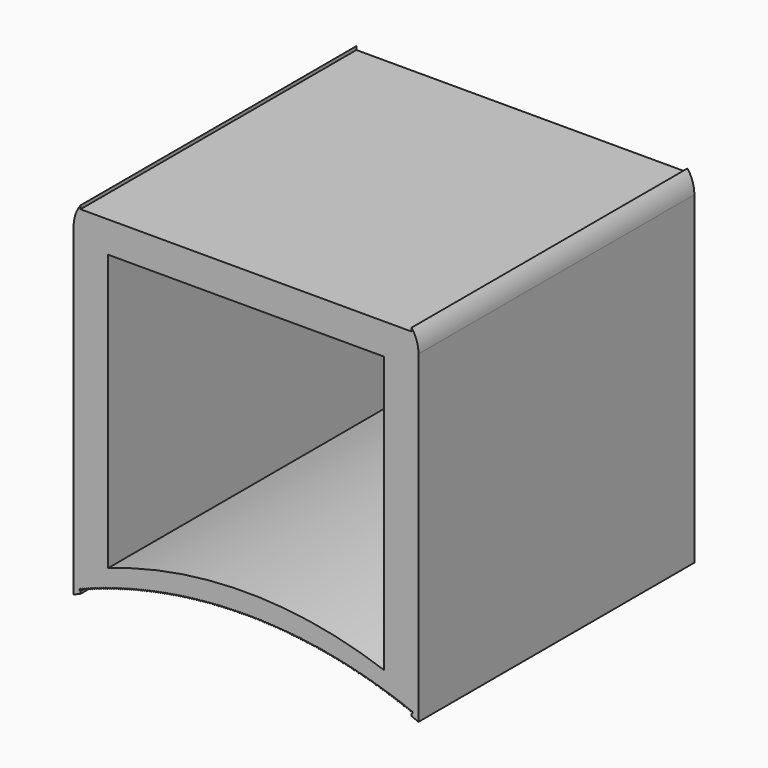
from build123d import *

# Parameters (mm, degrees)
F1_DEPTH    = 50
F2_W        = 48
F2_H        = 0.5
F2_H_2      = 1.5
F3_DEPTH    = 50
F4_T1_DEPTH = 65.1327459504
F6_DEPTH    = 50.001


# Not quite as in the source:
# - a fillet or chamfer that OpenCascade refuses, or shapes differently, is made with other operations: its cross-section is extruded or revolved along the edge and cut away or added


with BuildPart() as f1:
    # F0 (on Front) → F1 (new body)
    with BuildSketch(Plane.XZ):
        with BuildLine():
            Line((25, -25), (25, 25))
            Line((25, 25), (-25, 25))
            Line((-25, 25), (-25, -25))
            ThreePointArc((-25, -25), (0, -20), (25, -25))
        make_face()
        with BuildLine():
            Line((-20, 20), (20, 20))
            Line((20, 20), (20, -20))
            ThreePointArc((20, -20), (0, -16.5685424949), (-20, -20))
            Line((-20, -20), (-20, 20))
        make_face(mode=Mode.SUBTRACT)
    extrude(amount=F1_DEPTH)

    # F2 (on face) → F3 (cut)
    with BuildSketch(Plane.XZ.offset(50)):
        with Locations((0, 24.75)):
            Rectangle(F2_W, F2_H)
        with Locations((0, 25.75)):
            Rectangle(F2_W, F2_H_2)
        with BuildLine():
            Line((-24, -24.0930467578), (-24, -24.5930467578))
            ThreePointArc((-24, -24.5930467578), (0, -20), (24, -24.5930467578))
            Line((24, -24.5930467578), (24, -24.0930467578))
            ThreePointArc((24, -24.0930467578), (0, -19.5376937746), (-24, -24.0930467578))
        make_face()
    extrude(amount=-F3_DEPTH, mode=Mode.SUBTRACT)

    # F4: fillet of radius 5.08 on 2 edges, made by hand

    # F4_s2 → F4_t1 (cut)
    with BuildSketch(Plane.XZ.offset(-7.5663729752)):
        with BuildLine():
            ThreePointArc((25, 21.9734508099), (24.7435256815, 23.567188555), (24, 25))
            Line((24, 25), (25, 25))
            Line((25, 25), (25, 21.9734508099))
        make_face()
        with BuildLine():
            ThreePointArc((-25, 21.9734508099), (-24.7435256815, 23.567188555), (-24, 25))
            Line((-24, 25), (-25, 25))
            Line((-25, 25), (-25, 21.9734508099))
        make_face()
    extrude(amount=F4_T1_DEPTH, mode=Mode.SUBTRACT)

    # F5 (on face) → F6 (cut, through all)
    with BuildSketch(Plane.XZ.offset(50)):
        with BuildLine():
            ThreePointArc((-22.6266280663, -23.5699322866), (-22.8194734419, -23.4812633076), (-22.9079215474, -23.6742100862))
            ThreePointArc((-22.9079215474, -23.6742100862), (-22.7673345079, -23.6219101404), (-22.6266280663, -23.5699322866))
        make_face()
        with BuildLine():
            ThreePointArc((-22.9359440173, -23.6846785917), (-23.1292335577, -23.5969820679), (-23.2167087002, -23.7903718974))
            ThreePointArc((-23.2167087002, -23.7903718974), (-23.0763868702, -23.7373645013), (-22.9359440173, -23.6846785917))
        make_face()
        with BuildLine():
            ThreePointArc((-23.2446780865, -23.8009814147), (-23.438406888, -23.7142595708), (-23.5249068481, -23.908087545))
            ThreePointArc((-23.5249068481, -23.908087545), (-23.3848537877, -23.8543740434), (-23.2446780865, -23.8009814147))
        make_face()
        with BuildLine():
            ThreePointArc((-23.5528224413, -23.9188378049), (-23.7469855889, -23.833092841), (-23.8325081724, -24.0273540426))
            ThreePointArc((-23.8325081724, -24.0273540426), (-23.6927274345, -23.9729357982), (-23.5528224413, -23.9188378049))
        make_face()
        with BuildLine():
            ThreePointArc((-23.5528224413, -23.9188378049), (-23.6927274345, -23.9729357982), (-23.8325081724, -24.0273540426))
            ThreePointArc((-23.8325081724, -24.0273540426), (-23.6650426976, -24.1203588471), (-23.5427274345, -23.9729357982))
            ThreePointArc((-23.5427274345, -23.9729357982), (-23.5452727822, -23.9454198845), (-23.5528224413, -23.9188378049))
        make_face()
        with BuildLine():
            ThreePointArc((-23.2446780865, -23.8009814147), (-23.3848537877, -23.8543740434), (-23.5249068481, -23.908087545))
            ThreePointArc((-23.5249068481, -23.908087545), (-23.3575404125, -24.0018663467), (-23.2348537877, -23.8543740434))
            ThreePointArc((-23.2348537877, -23.8543740434), (-23.2373303062, -23.8272295705), (-23.2446780865, -23.8009814147))
        make_face()
        with BuildLine():
            ThreePointArc((-22.9359440173, -23.6846785917), (-23.0763868702, -23.7373645013), (-23.2167087002, -23.7903718974))
            ThreePointArc((-23.2167087002, -23.7903718974), (-23.04944503, -23.8849251236), (-22.9263868702, -23.7373645013))
            ThreePointArc((-22.9263868702, -23.7373645013), (-22.9287954952, -23.7105916413), (-22.9359440173, -23.6846785917))
        make_face()
        with BuildLine():
            ThreePointArc((-24, -24.2430467578), (-23.8939339828, -24.199112775), (-23.85, -24.0930467578))
            ThreePointArc((-23.85, -24.0930467578), (-23.8526151121, -24.0651595778), (-23.8603692642, -24.0382447724))
            ThreePointArc((-23.8603692642, -24.0382447724), (-23.9302003197, -24.0656057945), (-24, -24.0930467578))
            Line((-24, -24.0930467578), (-24, -24.2430467578))
        make_face()
        with BuildLine():
            ThreePointArc((-24, -24.0930467578), (-23.9302003197, -24.0656057945), (-23.8603692642, -24.0382447724))
            ThreePointArc((-23.8603692642, -24.0382447724), (-24.1239360678, -24.0085491183), (-24, -24.2430467578))
            Line((-24, -24.2430467578), (-24, -24.0930467578))
        make_face()
        with BuildLine():
            ThreePointArc((-19.8178993423, -22.6077260856), (-19.9608166732, -22.6532742635), (-20.1036293207, -22.6991496134))
            ThreePointArc((-20.1036293207, -22.6991496134), (-19.9375991919, -22.8014665324), (-19.8108166732, -22.6532742635))
            ThreePointArc((-19.8108166732, -22.6532742635), (-19.8125979166, -22.6302264832), (-19.8178993423, -22.6077260856))
        make_face()
        with BuildLine():
            ThreePointArc((-19.5031985114, -22.5086985178), (-19.6463434481, -22.553526267), (-19.7893853506, -22.5986817113))
            ThreePointArc((-19.7893853506, -22.5986817113), (-19.6234992516, -22.7017765375), (-19.4963434481, -22.553526267))
            ThreePointArc((-19.4963434481, -22.553526267), (-19.4980671174, -22.5308518376), (-19.5031985114, -22.5086985178))
        make_face()
        with BuildLine():
            ThreePointArc((-14.4061590265, -21.141586052), (-14.5857743357, -21.028493756), (-14.6986608912, -21.2082384424))
            ThreePointArc((-14.6986608912, -21.2082384424), (-14.5524481187, -21.1747447842), (-14.4061590265, -21.141586052))
        make_face()
        with BuildLine():
            ThreePointArc((-19.8178993423, -22.6077260856), (-20.0065284671, -22.5104091807), (-20.1036293207, -22.6991496134))
            ThreePointArc((-20.1036293207, -22.6991496134), (-19.9608166732, -22.6532742635), (-19.8178993423, -22.6077260856))
        make_face()
        with BuildLine():
            ThreePointArc((-19.188002887, -22.4112573024), (-19.3313717979, -22.4553634855), (-19.4746393264, -22.4997978786))
            ThreePointArc((-19.4746393264, -22.4997978786), (-19.308901031, -22.6036708172), (-19.1813717979, -22.4553634855))
            ThreePointArc((-19.1813717979, -22.4553634855), (-19.1830388335, -22.433062551), (-19.188002887, -22.4112573024))
        make_face()
        with BuildLine():
            ThreePointArc((-18.2395272787, -22.128476289), (-18.3835462664, -22.1704111336), (-18.5274688425, -22.2126756824))
            ThreePointArc((-18.5274688425, -22.2126756824), (-18.3621966342, -22.3188840038), (-18.2335462664, -22.1704111336))
            ThreePointArc((-18.2335462664, -22.1704111336), (-18.2350490473, -22.1492315225), (-18.2395272787, -22.128476289))
        make_face()
        with BuildLine():
            ThreePointArc((-12.7925832852, -20.7990775622), (-12.9396609786, -20.8285419833), (-13.0866708105, -20.8583431461))
            ThreePointArc((-13.0866708105, -20.8583431461), (-12.9246855787, -20.9777925692), (-12.7896609786, -20.8285419833))
            ThreePointArc((-12.7896609786, -20.8285419833), (-12.7903933431, -20.8137374908), (-12.7925832852, -20.7990775622))
        make_face()
        with BuildLine():
            ThreePointArc((-16.3302999565, -21.6060667789), (-16.5132505067, -21.4984534762), (-16.6206542534, -21.6815271277))
            ThreePointArc((-16.6206542534, -21.6815271277), (-16.4755203075, -21.6436307198), (-16.3302999565, -21.6060667789))
        make_face()
        with BuildLine():
            ThreePointArc((-17.2868871313, -21.8600590191), (-17.4315233127, -21.8998129502), (-17.5760680753, -21.9398980048))
            ThreePointArc((-17.5760680753, -21.9398980048), (-17.411296034, -22.0484428839), (-17.2815233127, -21.8998129502))
            ThreePointArc((-17.2815233127, -21.8998129502), (-17.2828703154, -21.8797558717), (-17.2868871313, -21.8600590191))
        make_face()
        with BuildLine():
            ThreePointArc((-16.9684525306, -21.7737892262), (-17.1132871112, -21.8128141445), (-17.2580319421, -21.8521706425))
            ThreePointArc((-17.2580319421, -21.8521706425), (-17.0934342101, -21.9614945477), (-16.9632871112, -21.8128141445))
            ThreePointArc((-16.9632871112, -21.8128141445), (-16.9645840731, -21.7931315011), (-16.9684525306, -21.7737892262))
        make_face()
        with BuildLine():
            ThreePointArc((-14.7278104328, -21.2149580149), (-14.8739306543, -21.2488531605), (-15.0199728701, -21.2830828435))
            ThreePointArc((-15.0199728701, -21.2830828435), (-14.8567017886, -21.3978604294), (-14.7239306543, -21.2488531605))
            ThreePointArc((-14.7239306543, -21.2488531605), (-14.7249037553, -21.2317949251), (-14.7278104328, -21.2149580149))
        make_face()
        with BuildLine():
            ThreePointArc((-21.0715952444, -23.0196490307), (-21.2621466389, -22.9261520106), (-21.3554254091, -23.1168103378))
            ThreePointArc((-21.3554254091, -23.1168103378), (-21.2135659535, -23.068067186), (-21.0715952444, -23.0196490307))
        make_face()
        with BuildLine():
            ThreePointArc((-22.0062819224, -23.3451208347), (-22.1982243024, -23.2545137187), (-22.2886115776, -23.4465597216))
            ThreePointArc((-22.2886115776, -23.4465597216), (-22.1475048257, -23.3956786389), (-22.0062819224, -23.3451208347))
        make_face()
        with BuildLine():
            ThreePointArc((-21.6952674677, -23.2350613913), (-21.8867510398, -23.1434886426), (-21.9781044725, -23.3350769436))
            ThreePointArc((-21.9781044725, -23.3350769436), (-21.8367432309, -23.2849072378), (-21.6952674677, -23.2350613913))
        make_face()
        with BuildLine():
            ThreePointArc((-20.4457847005, -22.8105301884), (-20.6353845803, -22.7151183848), (-20.7305792223, -22.9048273905))
            ThreePointArc((-20.7305792223, -22.9048273905), (-20.5882359484, -22.8575157391), (-20.4457847005, -22.8105301884))
        make_face()
        with BuildLine():
            ThreePointArc((-20.1320973957, -22.7083374933), (-20.321214297, -22.6119719166), (-20.4173632644, -22.8011990362))
            ThreePointArc((-20.4173632644, -22.8011990362), (-20.2747834951, -22.7546049444), (-20.1320973957, -22.7083374933))
        make_face()
        with BuildLine():
            ThreePointArc((-18.2395272787, -22.128476289), (-18.4256459906, -22.0264402573), (-18.5274688425, -22.2126756824))
            ThreePointArc((-18.5274688425, -22.2126756824), (-18.3835462664, -22.1704111336), (-18.2395272787, -22.128476289))
        make_face()
        with BuildLine():
            ThreePointArc((-13.1159803183, -20.8643265551), (-13.2932808097, -20.7476386703), (-13.4097656022, -20.9250726576))
            ThreePointArc((-13.4097656022, -20.9250726576), (-13.2629077386, -20.8945314086), (-13.1159803183, -20.8643265551))
        make_face()
        with BuildLine():
            ThreePointArc((-21.3837026069, -23.1265698725), (-21.5747225133, -23.0340338143), (-21.6670397858, -23.2251595528))
            ThreePointArc((-21.6670397858, -23.2251595528), (-21.5254276408, -23.1757024966), (-21.3837026069, -23.1265698725))
        make_face()
        with BuildLine():
            ThreePointArc((-14.4061590265, -21.141586052), (-14.5524481187, -21.1747447842), (-14.6986608912, -21.2082384424))
            ThreePointArc((-14.6986608912, -21.2082384424), (-14.5355945713, -21.3237949702), (-14.4024481187, -21.1747447842))
            ThreePointArc((-14.4024481187, -21.1747447842), (-14.4033787325, -21.1580619161), (-14.4061590265, -21.141586052))
        make_face()
        with BuildLine():
            ThreePointArc((-13.4390446008, -20.9312036179), (-13.6169305808, -20.8154102466), (-13.7325201899, -20.9934286978))
            ThreePointArc((-13.7325201899, -20.9934286978), (-13.5858180204, -20.9621481373), (-13.4390446008, -20.9312036179))
        make_face()
        with BuildLine():
            ThreePointArc((-14.7278104328, -21.2149580149), (-14.9079930909, -21.1027718461), (-15.0199728701, -21.2830828435))
            ThreePointArc((-15.0199728701, -21.2830828435), (-14.8739306543, -21.2488531605), (-14.7278104328, -21.2149580149))
        make_face()
        with BuildLine():
            ThreePointArc((-17.9224325672, -22.0374048001), (-18.1080349796, -21.9344326134), (-18.2107945769, -22.1201528113))
            ThreePointArc((-18.2107945769, -22.1201528113), (-18.0666609469, -22.0786137128), (-17.9224325672, -22.0374048001))
        make_face()
        with BuildLine():
            ThreePointArc((-18.5561592557, -22.2211437764), (-18.7427895454, -22.1200464882), (-18.8436730686, -22.3067924158))
            ThreePointArc((-18.8436730686, -22.3067924158), (-18.6999651977, -22.2638034889), (-18.5561592557, -22.2211437764))
        make_face()
        with BuildLine():
            ThreePointArc((-20.1320973957, -22.7083374933), (-20.2747834951, -22.7546049444), (-20.4173632644, -22.8011990362))
            ThreePointArc((-20.4173632644, -22.8011990362), (-20.2511928761, -22.9027382719), (-20.1247834951, -22.7546049444))
            ThreePointArc((-20.1247834951, -22.7546049444), (-20.1266232526, -22.7311839593), (-20.1320973957, -22.7083374933))
        make_face()
        with BuildLine():
            ThreePointArc((-15.0490881966, -21.2899491521), (-15.1950358402, -21.3245798512), (-15.3409037942, -21.3595446905))
            ThreePointArc((-15.3409037942, -21.3595446905), (-15.1774317654, -21.473543258), (-15.0450358402, -21.3245798512))
            ThreePointArc((-15.0450358402, -21.3245798512), (-15.0460523737, -21.3071463568), (-15.0490881966, -21.2899491521))
        make_face()
        with BuildLine():
            ThreePointArc((-13.7617679365, -20.9997070537), (-13.9402348921, -20.8848111336), (-14.0549263854, -21.0634095324))
            ThreePointArc((-14.0549263854, -21.0634095324), (-13.9083836318, -21.0313904542), (-13.7617679365, -20.9997070537))
        make_face()
        with BuildLine():
            ThreePointArc((-18.8723204655, -22.3154049114), (-19.0594575982, -22.2152489315), (-19.1593992332, -22.4025006239))
            ThreePointArc((-19.1593992332, -22.4025006239), (-19.0159097133, -22.3587884095), (-18.8723204655, -22.3154049114))
        make_face()
        with BuildLine():
            ThreePointArc((-19.5031985114, -22.5086985178), (-19.6913350743, -22.4104327536), (-19.7893853506, -22.5986817113))
            ThreePointArc((-19.7893853506, -22.5986817113), (-19.6463434481, -22.553526267), (-19.5031985114, -22.5086985178))
        make_face()
        with BuildLine():
            ThreePointArc((-12.7925832852, -20.7990775622), (-12.96929379, -20.6814981242), (-13.0866708105, -20.8583431461))
            ThreePointArc((-13.0866708105, -20.8583431461), (-12.9396609786, -20.8285419833), (-12.7925832852, -20.7990775622))
        make_face()
        with BuildLine():
            ThreePointArc((-14.0841421379, -21.0698351248), (-14.2305963894, -21.1022566024), (-14.3769760093, -21.1350133862))
            ThreePointArc((-14.3769760093, -21.1350133862), (-14.2141182673, -21.2513487601), (-14.0805963894, -21.1022566024))
            ThreePointArc((-14.0805963894, -21.1022566024), (-14.0814854614, -21.0859492073), (-14.0841421379, -21.0698351248))
        make_face()
        with BuildLine():
            ThreePointArc((-16.010598173, -21.5246183795), (-16.1560058853, -21.5614503931), (-16.3013288681, -21.5986153045))
            ThreePointArc((-16.3013288681, -21.5986153045), (-16.1372768628, -21.7102765457), (-16.0060058853, -21.5614503931))
            ThreePointArc((-16.0060058853, -21.5614503931), (-16.0071583847, -21.5428917945), (-16.010598173, -21.5246183795))
        make_face()
        with BuildLine():
            ThreePointArc((-21.0715952444, -23.0196490307), (-21.2135659535, -23.068067186), (-21.3554254091, -23.1168103378))
            ThreePointArc((-21.3554254091, -23.1168103378), (-21.1888568291, -23.2160180534), (-21.0635659535, -23.068067186))
            ThreePointArc((-21.0635659535, -23.068067186), (-21.0655868902, -23.0435274872), (-21.0715952444, -23.0196490307))
        make_face()
        with BuildLine():
            ThreePointArc((-17.6048831661, -21.9479316201), (-17.7899645702, -21.844025891), (-17.893658306, -22.0292261498))
            ThreePointArc((-17.893658306, -22.0292261498), (-17.7493172787, -21.9884135556), (-17.6048831661, -21.9479316201))
        make_face()
        with BuildLine():
            ThreePointArc((-13.7617679365, -20.9997070537), (-13.9083836318, -21.0313904542), (-14.0549263854, -21.0634095324))
            ThreePointArc((-14.0549263854, -21.0634095324), (-13.8922810395, -21.180523638), (-13.7583836318, -21.0313904542))
            ThreePointArc((-13.7583836318, -21.0313904542), (-13.7592321077, -21.0154586355), (-13.7617679365, -20.9997070537))
        make_face()
        with BuildLine():
            ThreePointArc((-18.8723204655, -22.3154049114), (-19.0159097133, -22.3587884095), (-19.1593992332, -22.4025006239))
            ThreePointArc((-19.1593992332, -22.4025006239), (-18.9938125187, -22.5071518618), (-18.8659097133, -22.3587884095))
            ThreePointArc((-18.8659097133, -22.3587884095), (-18.8675210561, -22.3368611111), (-18.8723204655, -22.3154049114))
        make_face()
        with BuildLine():
            ThreePointArc((-17.2868871313, -21.8600590191), (-17.4714428317, -21.7552223834), (-17.5760680753, -21.9398980048))
            ThreePointArc((-17.5760680753, -21.9398980048), (-17.4315233127, -21.8998129502), (-17.2868871313, -21.8600590191))
        make_face()
        with BuildLine():
            ThreePointArc((-13.4390446008, -20.9312036179), (-13.5858180204, -20.9621481373), (-13.7325201899, -20.9934286978))
            ThreePointArc((-13.7325201899, -20.9934286978), (-13.5700910599, -21.1113214014), (-13.4358180204, -20.9621481373))
            ThreePointArc((-13.4358180204, -20.9621481373), (-13.4366268462, -20.9465919962), (-13.4390446008, -20.9312036179))
        make_face()
        with BuildLine():
            ThreePointArc((-18.5561592557, -22.2211437764), (-18.6999651977, -22.2638034889), (-18.8436730686, -22.3067924158))
            ThreePointArc((-18.8436730686, -22.3067924158), (-18.6782417154, -22.4122221209), (-18.5499651977, -22.2638034889))
            ThreePointArc((-18.5499651977, -22.2638034889), (-18.5515217888, -22.2422499658), (-18.5561592557, -22.2211437764))
        make_face()
        with BuildLine():
            ThreePointArc((-16.9684525306, -21.7737892262), (-17.1524778451, -21.6680243438), (-17.2580319421, -21.8521706425))
            ThreePointArc((-17.2580319421, -21.8521706425), (-17.1132871112, -21.8128141445), (-16.9684525306, -21.7737892262))
        make_face()
        with BuildLine():
            ThreePointArc((-13.1159803183, -20.8643265551), (-13.2629077386, -20.8945314086), (-13.4097656022, -20.9250726576))
            ThreePointArc((-13.4097656022, -20.9250726576), (-13.2475565097, -21.0437438068), (-13.1129077386, -20.8945314086))
            ThreePointArc((-13.1129077386, -20.8945314086), (-13.1136778605, -20.8793510436), (-13.1159803183, -20.8643265551))
        make_face()
        with BuildLine():
            ThreePointArc((-16.6495874425, -21.6891244301), (-16.8330777024, -21.5824339842), (-16.9395579749, -21.7660462885))
            ThreePointArc((-16.9395579749, -21.7660462885), (-16.794616748, -21.7274193455), (-16.6495874425, -21.6891244301))
        make_face()
        with BuildLine():
            ThreePointArc((-17.9224325672, -22.0374048001), (-18.0666609469, -22.0786137128), (-18.2107945769, -22.1201528113))
            ThreePointArc((-18.2107945769, -22.1201528113), (-18.0456853004, -22.2271398797), (-17.9166609469, -22.0786137128))
            ThreePointArc((-17.9166609469, -22.0786137128), (-17.9181108595, -22.0578081481), (-17.9224325672, -22.0374048001))
        make_face()
        with BuildLine():
            ThreePointArc((-15.6904902028, -21.4447812985), (-15.8360815873, -21.4808804502), (-15.9815899203, -21.5173129223))
            ThreePointArc((-15.9815899203, -21.5173129223), (-15.8177274318, -21.6297532985), (-15.6860815873, -21.4808804502))
            ThreePointArc((-15.6860815873, -21.4808804502), (-15.6871878204, -21.4626967718), (-15.6904902028, -21.4447812985))
        make_face()
        with BuildLine():
            ThreePointArc((-17.6048831661, -21.9479316201), (-17.7493172787, -21.9884135556), (-17.893658306, -22.0292261498))
            ThreePointArc((-17.893658306, -22.0292261498), (-17.7287157508, -22.1369920771), (-17.5993172787, -21.9884135556))
            ThreePointArc((-17.5993172787, -21.9884135556), (-17.6007152651, -21.9679821692), (-17.6048831661, -21.9479316201))
        make_face()
        with BuildLine():
            ThreePointArc((-16.010598173, -21.5246183795), (-16.193004372, -21.4160849502), (-16.3013288681, -21.5986153045))
            ThreePointArc((-16.3013288681, -21.5986153045), (-16.1560058853, -21.5614503931), (-16.010598173, -21.5246183795))
        make_face()
        with BuildLine():
            ThreePointArc((-15.6904902028, -21.4447812985), (-15.872347423, -21.335330496), (-15.9815899203, -21.5173129223))
            ThreePointArc((-15.9815899203, -21.5173129223), (-15.8360815873, -21.4808804502), (-15.6904902028, -21.4447812985))
        make_face()
        with BuildLine():
            ThreePointArc((-20.4457847005, -22.8105301884), (-20.5882359484, -22.8575157391), (-20.7305792223, -22.9048273905))
            ThreePointArc((-20.7305792223, -22.9048273905), (-20.5642723415, -23.0055891855), (-20.4382359484, -22.8575157391))
            ThreePointArc((-20.4382359484, -22.8575157391), (-20.4401351597, -22.8337216977), (-20.4457847005, -22.8105301884))
        make_face()
        with BuildLine():
            ThreePointArc((-22.0062819224, -23.3451208347), (-22.1475048257, -23.3956786389), (-22.2886115776, -23.4465597216))
            ThreePointArc((-22.2886115776, -23.4465597216), (-22.1216786063, -23.543438601), (-21.9975048257, -23.3956786389))
            ThreePointArc((-21.9975048257, -23.3956786389), (-21.9997153885, -23.3700216272), (-22.0062819224, -23.3451208347))
        make_face()
        with BuildLine():
            ThreePointArc((-15.3699841669, -21.3665575612), (-15.5512877946, -21.2561921623), (-15.6614455217, -21.4376220438))
            ThreePointArc((-15.6614455217, -21.4376220438), (-15.5157555301, -21.4019229352), (-15.3699841669, -21.3665575612))
        make_face()
        with BuildLine():
            ThreePointArc((-16.6495874425, -21.6891244301), (-16.794616748, -21.7274193455), (-16.9395579749, -21.7660462885))
            ThreePointArc((-16.9395579749, -21.7660462885), (-16.7751383503, -21.8761492753), (-16.644616748, -21.7274193455))
            ThreePointArc((-16.644616748, -21.7274193455), (-16.6458646121, -21.708111262), (-16.6495874425, -21.6891244301))
        make_face()
        with BuildLine():
            ThreePointArc((-15.3699841669, -21.3665575612), (-15.5157555301, -21.4019229352), (-15.6614455217, -21.4376220438))
            ThreePointArc((-15.6614455217, -21.4376220438), (-15.4977763579, -21.550841535), (-15.3657555301, -21.4019229352))
            ThreePointArc((-15.3657555301, -21.4019229352), (-15.3668164411, -21.3841142923), (-15.3699841669, -21.3665575612))
        make_face()
        with BuildLine():
            ThreePointArc((-21.6952674677, -23.2350613913), (-21.8367432309, -23.2849072378), (-21.9781044725, -23.3350769436))
            ThreePointArc((-21.9781044725, -23.3350769436), (-21.8112892159, -23.4327317727), (-21.6867432309, -23.2849072378))
            ThreePointArc((-21.6867432309, -23.2849072378), (-21.6888896471, -23.2596225041), (-21.6952674677, -23.2350613913))
        make_face()
        with BuildLine():
            ThreePointArc((-15.0490881966, -21.2899491521), (-15.2298336322, -21.1786719567), (-15.3409037942, -21.3595446905))
            ThreePointArc((-15.3409037942, -21.3595446905), (-15.1950358402, -21.3245798512), (-15.0490881966, -21.2899491521))
        make_face()
        with BuildLine():
            ThreePointArc((-16.3302999565, -21.6060667789), (-16.4755203075, -21.6436307198), (-16.6206542534, -21.6815271277))
            ThreePointArc((-16.6206542534, -21.6815271277), (-16.4564165368, -21.7924092329), (-16.3255203075, -21.6436307198))
            ThreePointArc((-16.3255203075, -21.6436307198), (-16.3267200174, -21.6246973187), (-16.3302999565, -21.6060667789))
        make_face()
        with BuildLine():
            ThreePointArc((-21.3837026069, -23.1265698725), (-21.5254276408, -23.1757024966), (-21.6670397858, -23.2251595528))
            ThreePointArc((-21.6670397858, -23.2251595528), (-21.5003459916, -23.3235906668), (-21.3754276408, -23.1757024966))
            ThreePointArc((-21.3754276408, -23.1757024966), (-21.3775108482, -23.1507902014), (-21.3837026069, -23.1265698725))
        make_face()
        with BuildLine():
            ThreePointArc((-14.0841421379, -21.0698351248), (-14.2631855415, -20.9558395707), (-14.3769760093, -21.1350133862))
            ThreePointArc((-14.3769760093, -21.1350133862), (-14.2305963894, -21.1022566024), (-14.0841421379, -21.0698351248))
        make_face()
        with BuildLine():
            ThreePointArc((-19.188002887, -22.4112573024), (-19.375642115, -22.3120451719), (-19.4746393264, -22.4997978786))
            ThreePointArc((-19.4746393264, -22.4997978786), (-19.3313717979, -22.4553634855), (-19.188002887, -22.4112573024))
        make_face()
        with BuildLine():
            ThreePointArc((-20.7589532984, -22.9143015785), (-20.9490313467, -22.8198459684), (-21.0432692482, -23.0100320474))
            ThreePointArc((-21.0432692482, -23.0100320474), (-20.9011660808, -22.9620040365), (-20.7589532984, -22.9143015785))
        make_face()
        with BuildLine():
            ThreePointArc((-20.7589532984, -22.9143015785), (-20.9011660808, -22.9620040365), (-21.0432692482, -23.0100320474))
            ThreePointArc((-21.0432692482, -23.0100320474), (-20.876829638, -23.1100166628), (-20.7511660808, -22.9620040365))
            ThreePointArc((-20.7511660808, -22.9620040365), (-20.7531256854, -22.9378370898), (-20.7589532984, -22.9143015785))
        make_face()
        with BuildLine():
            ThreePointArc((-22.3167380807, -23.4567454104), (-22.509134399, -23.3671062259), (-22.5985532236, -23.5596050584))
            ThreePointArc((-22.5985532236, -23.5596050584), (-22.4577045413, -23.5080138897), (-22.3167380807, -23.4567454104))
        make_face()
        with BuildLine():
            ThreePointArc((-22.6266280663, -23.5699322866), (-22.7673345079, -23.6219101404), (-22.9079215474, -23.6742100862))
            ThreePointArc((-22.9079215474, -23.6742100862), (-22.7407643735, -23.7695381457), (-22.6173345079, -23.6219101404))
            ThreePointArc((-22.6173345079, -23.6219101404), (-22.6196761755, -23.5955090632), (-22.6266280663, -23.5699322866))
        make_face()
        with BuildLine():
            ThreePointArc((-22.3167380807, -23.4567454104), (-22.4577045413, -23.5080138897), (-22.5985532236, -23.5596050584))
            ThreePointArc((-22.5985532236, -23.5596050584), (-22.4315062813, -23.6557083418), (-22.3077045413, -23.5080138897))
            ThreePointArc((-22.3077045413, -23.5080138897), (-22.309980188, -23.4819847627), (-22.3167380807, -23.4567454104))
        make_face()
        with BuildLine():
            ThreePointArc((-4.2944910455, -19.6786290119), (-4.4543343924, -19.5389807711), (-4.593799515, -19.6989839158))
            ThreePointArc((-4.593799515, -19.6989839158), (-4.4441569338, -19.6886351039), (-4.2944910455, -19.6786290119))
        make_face()
        with BuildLine():
            ThreePointArc((-4.6236393908, -19.7010887298), (-4.7841840952, -19.562247365), (-4.9228415392, -19.7229509429))
            ThreePointArc((-4.9228415392, -19.7229509429), (-4.7732529815, -19.7118485373), (-4.6236393908, -19.7010887298))
        make_face()
        with BuildLine():
            ThreePointArc((-4.9526704349, -19.7252060287), (-5.1139124239, -19.5871750622), (-5.2517586717, -19.7485749963))
            ThreePointArc((-5.2517586717, -19.7485749963), (-5.1022279325, -19.7367192786), (-4.9526704349, -19.7252060287))
        make_face()
        with BuildLine():
            ThreePointArc((-9.5421205759, -20.2364751525), (-9.6904951943, -20.258497246), (-9.8388189914, -20.2808590708))
            ThreePointArc((-9.8388189914, -20.2808590708), (-9.6792829146, -20.4080776083), (-9.5404951943, -20.258497246))
            ThreePointArc((-9.5404951943, -20.258497246), (-9.5409020916, -20.2474562489), (-9.5421205759, -20.2364751525))
        make_face()
        with BuildLine():
            ThreePointArc((-9.2156064931, -20.1892350654), (-9.3855346323, -20.0620503406), (-9.5125246995, -20.2321239998))
            ThreePointArc((-9.5125246995, -20.2321239998), (-9.364090151, -20.2105095411), (-9.2156064931, -20.1892350654))
        make_face()
        with BuildLine():
            ThreePointArc((-7.9072950985, -20.0167380432), (-8.074626479, -19.8861557481), (-8.2050170878, -20.0536365406))
            ThreePointArc((-8.2050170878, -20.0536365406), (-8.0561772182, -20.0350168403), (-7.9072950985, -20.0167380432))
        make_face()
        with BuildLine():
            ThreePointArc((-9.5421205759, -20.2364751525), (-9.712687168, -20.110147941), (-9.8388189914, -20.2808590708))
            ThreePointArc((-9.8388189914, -20.2808590708), (-9.6904951943, -20.258497246), (-9.5421205759, -20.2364751525))
        make_face()
        with BuildLine():
            ThreePointArc((-8.2346946162, -20.0573905699), (-8.4026815956, -19.9276527517), (-8.5322269772, -20.0957881758))
            ThreePointArc((-8.5322269772, -20.0957881758), (-8.3834827801, -20.0764190298), (-8.2346946162, -20.0573905699))
        make_face()
        with BuildLine():
            ThreePointArc((-9.8683925764, -20.2853592379), (-10.0166543911, -20.3081283906), (-10.1648636739, -20.3312370142))
            ThreePointArc((-10.1648636739, -20.3312370142), (-10.0050654399, -20.4576800412), (-9.8666543911, -20.3081283906))
            ThreePointArc((-9.8666543911, -20.3081283906), (-9.8670895687, -20.2967106894), (-9.8683925764, -20.2853592379))
        make_face()
        with BuildLine():
            ThreePointArc((-8.5618852208, -20.0996916382), (-8.7305235373, -19.9708015885), (-8.8592204053, -20.1395873784))
            ThreePointArc((-8.8592204053, -20.1395873784), (-8.7105756541, -20.1194692782), (-8.5618852208, -20.0996916382))
        make_face()
        with BuildLine():
            ThreePointArc((-7.5796949738, -19.9777350895), (-7.7463665103, -19.8463116303), (-7.8775990381, -20.0131335424))
            ThreePointArc((-7.8775990381, -20.0131335424), (-7.7286672722, -19.9952637601), (-7.5796949738, -19.9777350895))
        make_face()
        with BuildLine():
            ThreePointArc((-8.8888586115, -20.143640175), (-9.037447542, -20.1641664933), (-9.185989076, -20.1850330374))
            ThreePointArc((-9.185989076, -20.1850330374), (-9.0269888161, -20.3138014325), (-8.887447542, -20.1641664933))
            ThreePointArc((-8.887447542, -20.1641664933), (-8.8878007252, -20.153879112), (-8.8888586115, -20.143640175))
        make_face()
        with BuildLine():
            ThreePointArc((-10.8456733411, -20.4418628737), (-10.9935741881, -20.4668696621), (-11.1414173798, -20.4922150889))
            ThreePointArc((-11.1414173798, -20.4922150889), (-10.9808556732, -20.6163294874), (-10.8435741881, -20.4668696621))
            ThreePointArc((-10.8435741881, -20.4668696621), (-10.8440998976, -20.4543222928), (-10.8456733411, -20.4418628737))
        make_face()
        with BuildLine():
            ThreePointArc((-12.4688617059, -20.7354582944), (-12.6449777409, -20.6169902863), (-12.7632440117, -20.7932418562))
            ThreePointArc((-12.7632440117, -20.7932418562), (-12.616085941, -20.7641815357), (-12.4688617059, -20.7354582944))
        make_face()
        with BuildLine():
            ThreePointArc((-8.5618852208, -20.0996916382), (-8.7105756541, -20.1194692782), (-8.8592204053, -20.1395873784))
            ThreePointArc((-8.8592204053, -20.1395873784), (-8.7004938058, -20.2691300824), (-8.5605756541, -20.1194692782))
            ThreePointArc((-8.5605756541, -20.1194692782), (-8.5609034039, -20.1095588038), (-8.5618852208, -20.0996916382))
        make_face()
        with BuildLine():
            ThreePointArc((-12.1448237933, -20.6734703657), (-12.3203408905, -20.554116793), (-12.4394934112, -20.7297704395))
            ThreePointArc((-12.4394934112, -20.7297704395), (-12.2921908351, -20.7014516985), (-12.1448237933, -20.6734703657))
        make_face()
        with BuildLine():
            ThreePointArc((-11.8204777681, -20.6131153489), (-11.9953914746, -20.4928792395), (-12.1154272223, -20.6679305063))
            ThreePointArc((-12.1154272223, -20.6679305063), (-11.9679838779, -20.6403540633), (-11.8204777681, -20.6131153489))
        make_face()
        with BuildLine():
            ThreePointArc((-7.9072950985, -20.0167380432), (-8.0561772182, -20.0350168403), (-8.2050170878, -20.0536365406))
            ThreePointArc((-8.2050170878, -20.0536365406), (-8.0468493146, -20.1847265267), (-7.9061772182, -20.0350168403))
            ThreePointArc((-7.9061772182, -20.0350168403), (-7.9064569491, -20.0258603661), (-7.9072950985, -20.0167380432))
        make_face()
        with BuildLine():
            ThreePointArc((-6.2674546999, -19.8382381666), (-6.4314447449, -19.703483605), (-6.5660114433, -19.8676278415))
            ThreePointArc((-6.5660114433, -19.8676278415), (-6.4167498978, -19.8527620745), (-6.2674546999, -19.8382381666))
        make_face()
        with BuildLine():
            ThreePointArc((-11.495831859, -20.554394775), (-11.6701377373, -20.4332791794), (-11.7910536666, -20.6077236254))
            ThreePointArc((-11.7910536666, -20.6077236254), (-11.6434732946, -20.58089018), (-11.495831859, -20.554394775))
        make_face()
        with BuildLine():
            ThreePointArc((-7.5796949738, -19.9777350895), (-7.7286672722, -19.9952637601), (-7.8775990381, -20.0131335424))
            ThreePointArc((-7.8775990381, -20.0131335424), (-7.7197164309, -20.1449964634), (-7.5786672722, -19.9952637601))
            ThreePointArc((-7.5786672722, -19.9952637601), (-7.578924418, -19.9864843743), (-7.5796949738, -19.9777350895))
        make_face()
        with BuildLine():
            ThreePointArc((-12.4688617059, -20.7354582944), (-12.616085941, -20.7641815357), (-12.7632440117, -20.7932418562))
            ThreePointArc((-12.7632440117, -20.7932418562), (-12.6014864651, -20.9134693627), (-12.466085941, -20.7641815357))
            ThreePointArc((-12.466085941, -20.7641815357), (-12.4667814949, -20.7497530096), (-12.4688617059, -20.7354582944))
        make_face()
        with BuildLine():
            ThreePointArc((-5.9389763021, -19.8074970826), (-6.1022855303, -19.6719182395), (-6.2376772892, -19.8353826037))
            ThreePointArc((-6.2376772892, -19.8353826037), (-6.0883427606, -19.821268831), (-5.9389763021, -19.8074970826))
        make_face()
        with BuildLine():
            ThreePointArc((-11.1708943021, -20.4973101339), (-11.3445879301, -20.3753181247), (-11.4663809735, -20.5491513243))
            ThreePointArc((-11.4663809735, -20.5491513243), (-11.3186673179, -20.5230615572), (-11.1708943021, -20.4973101339))
        make_face()
        with BuildLine():
            ThreePointArc((-12.1448237933, -20.6734703657), (-12.2921908351, -20.7014516985), (-12.4394934112, -20.7297704395))
            ThreePointArc((-12.4394934112, -20.7297704395), (-12.2779673757, -20.8507758198), (-12.1421908351, -20.7014516985))
            ThreePointArc((-12.1421908351, -20.7014516985), (-12.1428505253, -20.6873992303), (-12.1448237933, -20.6734703657))
        make_face()
        with BuildLine():
            ThreePointArc((-5.6103472332, -19.77841088), (-5.7729715016, -19.6420111951), (-5.9091848861, -19.8047915398))
            ThreePointArc((-5.9091848861, -19.8047915398), (-5.759781163, -19.7914301195), (-5.6103472332, -19.77841088))
        make_face()
        with BuildLine():
            ThreePointArc((-10.8456733411, -20.4418628737), (-11.0187503122, -20.3189975458), (-11.1414173798, -20.4922150889))
            ThreePointArc((-11.1414173798, -20.4922150889), (-10.9935741881, -20.4668696621), (-10.8456733411, -20.4418628737))
        make_face()
        with BuildLine():
            ThreePointArc((-5.2815758305, -19.7509802967), (-5.4435110133, -19.6137632305), (-5.5805425677, -19.7758554259))
            ThreePointArc((-5.5805425677, -19.7758554259), (-5.4310734406, -19.763246697), (-5.2815758305, -19.7509802967))
        make_face()
        with BuildLine():
            ThreePointArc((-10.5201772268, -20.3880544012), (-10.6926331501, -20.2643188717), (-10.8161711298, -20.4369163637))
            ThreePointArc((-10.8161711298, -20.4369163637), (-10.6682021528, -20.4123159202), (-10.5201772268, -20.3880544012))
        make_face()
        with BuildLine():
            ThreePointArc((-11.8204777681, -20.6131153489), (-11.9679838779, -20.6403540633), (-12.1154272223, -20.6679305063))
            ThreePointArc((-12.1154272223, -20.6679305063), (-11.9541365253, -20.7897135318), (-11.8179838779, -20.6403540633))
            ThreePointArc((-11.8179838779, -20.6403540633), (-11.8186086516, -20.6266777421), (-11.8204777681, -20.6131153489))
        make_face()
        with BuildLine():
            ThreePointArc((-10.1944142171, -20.3358860814), (-10.3662447173, -20.2112834895), (-10.4906504751, -20.3832565517))
            ThreePointArc((-10.4906504751, -20.3832565517), (-10.3425594666, -20.3594017155), (-10.1944142171, -20.3358860814))
        make_face()
        with BuildLine():
            ThreePointArc((-10.1944142171, -20.3358860814), (-10.3425594666, -20.3594017155), (-10.4906504751, -20.3832565517))
            ThreePointArc((-10.4906504751, -20.3832565517), (-10.3305939175, -20.508923706), (-10.1925594666, -20.3594017155))
            ThreePointArc((-10.1925594666, -20.3594017155), (-10.1930238731, -20.3476073827), (-10.1944142171, -20.3358860814))
        make_face()
        with BuildLine():
            ThreePointArc((-6.2674546999, -19.8382381666), (-6.4167498978, -19.8527620745), (-6.5660114433, -19.8676278415))
            ThreePointArc((-6.5660114433, -19.8676278415), (-6.4093078493, -20.0025773471), (-6.2667498978, -19.8527620745))
            ThreePointArc((-6.2667498978, -19.8527620745), (-6.2669262019, -19.8454915751), (-6.2674546999, -19.8382381666))
        make_face()
        with BuildLine():
            ThreePointArc((-9.8683925764, -20.2853592379), (-10.0395932942, -20.1598927446), (-10.1648636739, -20.3312370142))
            ThreePointArc((-10.1648636739, -20.3312370142), (-10.0166543911, -20.3081283906), (-9.8683925764, -20.2853592379))
        make_face()
        with BuildLine():
            ThreePointArc((-11.1708943021, -20.4973101339), (-11.3186673179, -20.5230615572), (-11.4663809735, -20.5491513243))
            ThreePointArc((-11.4663809735, -20.5491513243), (-11.3055724399, -20.6724888779), (-11.1686673179, -20.5230615572))
            ThreePointArc((-11.1686673179, -20.5230615572), (-11.169225101, -20.5101377878), (-11.1708943021, -20.4973101339))
        make_face()
        with BuildLine():
            ThreePointArc((-8.8888586115, -20.143640175), (-9.0581439867, -20.0156011636), (-9.185989076, -20.1850330374))
            ThreePointArc((-9.185989076, -20.1850330374), (-9.037447542, -20.1641664933), (-8.8888586115, -20.143640175))
        make_face()
        with BuildLine():
            ThreePointArc((-5.9389763021, -19.8074970826), (-6.0883427606, -19.821268831), (-6.2376772892, -19.8353826037))
            ThreePointArc((-6.2376772892, -19.8353826037), (-6.0812780343, -19.9711023708), (-5.9383427606, -19.821268831))
            ThreePointArc((-5.9383427606, -19.821268831), (-5.9385012297, -19.8143756744), (-5.9389763021, -19.8074970826))
        make_face()
        with BuildLine():
            ThreePointArc((-9.2156064931, -20.1892350654), (-9.364090151, -20.2105095411), (-9.5125246995, -20.2321239998))
            ThreePointArc((-9.5125246995, -20.2321239998), (-9.3532546139, -20.3601176664), (-9.214090151, -20.2105095411))
            ThreePointArc((-9.214090151, -20.2105095411), (-9.2144697168, -20.1998453181), (-9.2156064931, -20.1892350654))
        make_face()
        with BuildLine():
            ThreePointArc((-5.6103472332, -19.77841088), (-5.759781163, -19.7914301195), (-5.9091848861, -19.8047915398))
            ThreePointArc((-5.9091848861, -19.8047915398), (-5.7530938037, -19.9412809761), (-5.609781163, -19.7914301195))
            ThreePointArc((-5.609781163, -19.7914301195), (-5.6099227474, -19.7849143495), (-5.6103472332, -19.77841088))
        make_face()
        with BuildLine():
            ThreePointArc((-7.2519025532, -19.9403826984), (-7.4179100172, -19.8081214092), (-7.5499811348, -19.9742802086))
            ThreePointArc((-7.5499811348, -19.9742802086), (-7.400961251, -19.9571607977), (-7.2519025532, -19.9403826984))
        make_face()
        with BuildLine():
            ThreePointArc((-6.9239261528, -19.9046818173), (-7.0892653327, -19.7715860537), (-7.2221716894, -19.9370775249))
            ThreePointArc((-7.2221716894, -19.9370775249), (-7.0730674683, -19.9207089198), (-6.9239261528, -19.9046818173))
        make_face()
        with BuildLine():
            ThreePointArc((-8.2346946162, -20.0573905699), (-8.3834827801, -20.0764190298), (-8.5322269772, -20.0957881758))
            ThreePointArc((-8.5322269772, -20.0957881758), (-8.3737778734, -20.2261047498), (-8.2334827801, -20.0764190298))
            ThreePointArc((-8.2334827801, -20.0764190298), (-8.2337860457, -20.0668855253), (-8.2346946162, -20.0573905699))
        make_face()
        with BuildLine():
            ThreePointArc((-6.5957740933, -19.8706333521), (-6.7604407945, -19.7367064906), (-6.8941790186, -19.9015264353))
            ThreePointArc((-6.8941790186, -19.9015264353), (-6.7449942428, -19.8859090511), (-6.5957740933, -19.8706333521))
        make_face()
        with BuildLine():
            ThreePointArc((-5.2815758305, -19.7509802967), (-5.4310734406, -19.763246697), (-5.5805425677, -19.7758554259))
            ThreePointArc((-5.5805425677, -19.7758554259), (-5.4247634907, -19.9131139201), (-5.2810734406, -19.763246697))
            ThreePointArc((-5.2810734406, -19.763246697), (-5.2811990907, -19.757108355), (-5.2815758305, -19.7509802967))
        make_face()
        with BuildLine():
            ThreePointArc((-10.5201772268, -20.3880544012), (-10.6682021528, -20.4123159202), (-10.8161711298, -20.4369163637))
            ThreePointArc((-10.8161711298, -20.4369163637), (-10.6558600817, -20.5618073022), (-10.5182021528, -20.4123159202))
            ThreePointArc((-10.5182021528, -20.4123159202), (-10.5186967367, -20.4001450305), (-10.5201772268, -20.3880544012))
        make_face()
        with BuildLine():
            ThreePointArc((-7.2519025532, -19.9403826984), (-7.400961251, -19.9571607977), (-7.5499811348, -19.9742802086))
            ThreePointArc((-7.5499811348, -19.9742802086), (-7.3923875287, -20.1069155682), (-7.250961251, -19.9571607977))
            ThreePointArc((-7.250961251, -19.9571607977), (-7.2511967614, -19.9487585559), (-7.2519025532, -19.9403826984))
        make_face()
        with BuildLine():
            ThreePointArc((-6.5957740933, -19.8706333521), (-6.7449942428, -19.8859090511), (-6.8941790186, -19.9015264353))
            ThreePointArc((-6.8941790186, -19.9015264353), (-6.7371749193, -20.0357051064), (-6.5949942428, -19.8859090511))
            ThreePointArc((-6.5949942428, -19.8859090511), (-6.5951893323, -19.8782612549), (-6.5957740933, -19.8706333521))
        make_face()
        with BuildLine():
            ThreePointArc((-11.495831859, -20.554394775), (-11.6434732946, -20.58089018), (-11.7910536666, -20.6077236254))
            ThreePointArc((-11.7910536666, -20.6077236254), (-11.6300021366, -20.7302840483), (-11.4934732946, -20.58089018))
            ThreePointArc((-11.4934732946, -20.58089018), (-11.4940640992, -20.5675900925), (-11.495831859, -20.554394775))
        make_face()
        with BuildLine():
            ThreePointArc((-6.9239261528, -19.9046818173), (-7.0730674683, -19.9207089198), (-7.2221716894, -19.9370775249))
            ThreePointArc((-7.2221716894, -19.9370775249), (-7.0648709194, -20.0704848076), (-6.9230674683, -19.9207089198))
            ThreePointArc((-6.9230674683, -19.9207089198), (-6.9232822933, -19.9126838753), (-6.9239261528, -19.9046818173))
        make_face()
        with BuildLine():
            ThreePointArc((7.5921431638, -19.9791865509), (7.7411121057, -19.9967437249), (7.8900404497, -20.0146420029))
            ThreePointArc((7.8900404497, -20.0146420029), (7.890843952, -20.0057088909), (7.8911121057, -19.9967437249))
            ThreePointArc((7.8911121057, -19.9967437249), (7.7499058171, -19.8470017113), (7.5921431638, -19.9791865509))
        make_face()
        with BuildLine():
            ThreePointArc((11.5081696414, -20.5565955248), (11.6558060048, -20.5831191784), (11.8033812399, -20.6099808608))
            ThreePointArc((11.8033812399, -20.6099808608), (11.8051985837, -20.5966046286), (11.8058060048, -20.5831191784))
            ThreePointArc((11.8058060048, -20.5831191784), (11.669120386, -20.4337112561), (11.5081696414, -20.5565955248))
        make_face()
        with BuildLine():
            ThreePointArc((9.8807818649, -20.2872486044), (10.0290393203, -20.3100461246), (10.1772441789, -20.3331831056))
            ThreePointArc((10.1772441789, -20.3331831056), (10.1785898616, -20.321649383), (10.1790393203, -20.3100461246))
            ThreePointArc((10.1790393203, -20.3100461246), (10.04047133, -20.1604823951), (9.8807818649, -20.2872486044))
        make_face()
        with BuildLine():
            ThreePointArc((7.9197358199, -20.0182521856), (8.0501366965, -20.1854170284), (8.2174507437, -20.0552076474))
            ThreePointArc((8.2174507437, -20.0552076474), (8.0686144395, -20.0365594689), (7.9197358199, -20.0182521856))
        make_face()
        with BuildLine():
            ThreePointArc((-4.9526704349, -19.7252060287), (-5.1022279325, -19.7367192786), (-5.2517586717, -19.7485749963))
            ThreePointArc((-5.2517586717, -19.7485749963), (-5.096295432, -19.8866019175), (-4.9522279325, -19.7367192786))
            ThreePointArc((-4.9522279325, -19.7367192786), (-4.9523385989, -19.7309584034), (-4.9526704349, -19.7252060287))
        make_face()
        with BuildLine():
            ThreePointArc((10.206793832, -20.3378378268), (10.3549345794, -20.3613818061), (10.5030210209, -20.385264977))
            ThreePointArc((10.5030210209, -20.385264977), (10.5044554245, -20.3733616596), (10.5049345794, -20.3613818061))
            ThreePointArc((10.5049345794, -20.3613818061), (10.366743218, -20.2118473416), (10.206793832, -20.3378378268))
        make_face()
        with BuildLine():
            ThreePointArc((4.965166991, -19.7261548496), (5.1030091785, -19.8872386931), (5.264250751, -19.7495810432))
            ThreePointArc((5.264250751, -19.7495810432), (5.114722283, -19.7376967151), (4.965166991, -19.7261548496))
        make_face()
        with BuildLine():
            ThreePointArc((0.9810291731, -19.5429658149), (0.8318948761, -19.3929683131), (0.6810391657, -19.5412344378))
            ThreePointArc((0.6810391657, -19.5412344378), (0.8310291731, -19.5429658149), (0.9810148223, -19.5450406758))
            ThreePointArc((0.9810148223, -19.5450406758), (0.9810255854, -19.5440032702), (0.9810291731, -19.5429658149))
        make_face()
        with BuildLine():
            ThreePointArc((7.2643578961, -19.9417714418), (7.4134133809, -19.9585780612), (7.5624299864, -19.9757259847))
            ThreePointArc((7.5624299864, -19.9757259847), (7.5631673305, -19.9671661102), (7.5634133809, -19.9585780612))
            ThreePointArc((7.5634133809, -19.9585780612), (7.4218299503, -19.8088143761), (7.2643578961, -19.9417714418))
        make_face()
        with BuildLine():
            ThreePointArc((-4.2944910455, -19.6786290119), (-4.4441569338, -19.6886351039), (-4.593799515, -19.6989839158))
            ThreePointArc((-4.593799515, -19.6989839158), (-4.4389794427, -19.8385457226), (-4.2941569338, -19.6886351039))
            ThreePointArc((-4.2941569338, -19.6886351039), (-4.294240485, -19.6836292696), (-4.2944910455, -19.6786290119))
        make_face()
        with BuildLine():
            ThreePointArc((11.1832430129, -20.4994487124), (11.3310110988, -20.5252284096), (11.4787197598, -20.5513464391))
            ThreePointArc((11.4787197598, -20.5513464391), (11.480437166, -20.5383375829), (11.4810110988, -20.5252284096))
            ThreePointArc((11.4810110988, -20.5252284096), (11.343949165, -20.3757874298), (11.1832430129, -20.4994487124))
        make_face()
        with BuildLine():
            ThreePointArc((0.9810148223, -19.5450406758), (0.8310291731, -19.5429658149), (0.6810391657, -19.5412344378))
            ThreePointArc((0.6810391657, -19.5412344378), (0.8291260529, -19.6929537416), (0.9810148223, -19.5450406758))
        make_face()
        with BuildLine():
            ThreePointArc((-2.6472821605, -19.5912126075), (-2.8035582511, -19.4475835359), (-2.9470082865, -19.6040239848))
            ThreePointArc((-2.9470082865, -19.6040239848), (-2.7971525582, -19.5974466971), (-2.6472821605, -19.5912126075))
        make_face()
        with BuildLine():
            ThreePointArc((-3.9652337496, -19.6578274448), (-4.1243716838, -19.5173758708), (-4.2646409466, -19.6766745231))
            ThreePointArc((-4.2646409466, -19.6766745231), (-4.1149481384, -19.6670795675), (-3.9652337496, -19.6578274448))
        make_face()
        with BuildLine():
            ThreePointArc((-2.9768917025, -19.605376715), (-3.1338892467, -19.4625366022), (-3.2765494977, -19.6196976009))
            ThreePointArc((-3.2765494977, -19.6196976009), (-3.1267287991, -19.612365598), (-2.9768917025, -19.605376715))
        make_face()
        with BuildLine():
            ThreePointArc((-3.9652337496, -19.6578274448), (-4.1149481384, -19.6670795675), (-4.2646409466, -19.6766745231))
            ThreePointArc((-4.2646409466, -19.6766745231), (-4.1101482025, -19.8170027499), (-3.9649481384, -19.6670795675))
            ThreePointArc((-3.9649481384, -19.6670795675), (-3.9650195582, -19.6624513025), (-3.9652337496, -19.6578274448))
        make_face()
        with BuildLine():
            ThreePointArc((6.2799296048, -19.8394385514), (6.4144986118, -20.0032666797), (6.5784807194, -19.8688853505))
            ThreePointArc((6.5784807194, -19.8688853505), (6.429222021, -19.8539910246), (6.2799296048, -19.8394385514))
        make_face()
        with BuildLine():
            ThreePointArc((1.0109253811, -19.5454955379), (1.1582462048, -19.6979588063), (1.3108780612, -19.5508126555))
            ThreePointArc((1.3108780612, -19.5508126555), (1.1609047653, -19.547982368), (1.0109253811, -19.5454955379))
        make_face()
        with BuildLine():
            ThreePointArc((0.6511266952, -19.5409302361), (0.5011324979, -19.5396108544), (0.3511356724, -19.5386349742))
            ThreePointArc((0.3511356724, -19.5386349742), (0.4999848662, -19.6896064642), (0.6511266952, -19.5409302361))
        make_face()
        with BuildLine():
            ThreePointArc((5.6228335972, -19.7794855374), (5.7590461058, -19.9419497667), (5.9216661971, -19.8059233751))
            ThreePointArc((5.9216661971, -19.8059233751), (5.7722650333, -19.7925333688), (5.6228335972, -19.7794855374))
        make_face()
        with BuildLine():
            ThreePointArc((10.8580326669, -20.4439392266), (11.0059287265, -20.4689743134), (11.153767066, -20.4943480275))
            ThreePointArc((11.153767066, -20.4943480275), (11.1553873343, -20.4817071267), (11.1559287265, -20.4689743134))
            ThreePointArc((11.1559287265, -20.4689743134), (11.0184903957, -20.3195012239), (10.8580326669, -20.4439392266))
        make_face()
        with BuildLine():
            ThreePointArc((-4.6236393908, -19.7010887298), (-4.7732529815, -19.7118485373), (-4.9228415392, -19.7229509429))
            ThreePointArc((-4.9228415392, -19.7229509429), (-4.7676979682, -19.8617456414), (-4.6232529815, -19.7118485373))
            ThreePointArc((-4.6232529815, -19.7118485373), (-4.623349615, -19.7064651654), (-4.6236393908, -19.7010887298))
        make_face()
        with BuildLine():
            ThreePointArc((6.9363883326, -19.9060078077), (7.0855265788, -19.9220634459), (7.2346276653, -19.9384605799))
            ThreePointArc((7.2346276653, -19.9384605799), (7.2353016818, -19.9302743236), (7.2355265788, -19.9220634459))
            ThreePointArc((7.2355265788, -19.9220634459), (7.0935659529, -19.7722790393), (6.9363883326, -19.9060078077))
        make_face()
        with BuildLine():
            ThreePointArc((-3.3064257211, -19.6212008317), (-3.4641407359, -19.4791533015), (-3.6060075833, -19.6370308628))
            ThreePointArc((-3.6060075833, -19.6370308628), (-3.4562257152, -19.6289443308), (-3.3064257211, -19.6212008317))
        make_face()
        with BuildLine():
            ThreePointArc((1.0109253811, -19.5454955379), (1.1609047653, -19.547982368), (1.3108780612, -19.5508126555))
            ThreePointArc((1.3108780612, -19.5508126555), (1.3108980891, -19.5493975747), (1.3109047653, -19.547982368))
            ThreePointArc((1.3109047653, -19.547982368), (1.1621482231, -19.397987522), (1.0109253811, -19.5454955379))
        make_face()
        with BuildLine():
            ThreePointArc((-0.0086907464, -19.5376943512), (-0.1586906239, -19.5378860094), (-0.3086896692, -19.538421178))
            ThreePointArc((-0.3086896692, -19.538421178), (-0.1584230392, -19.6878857707), (-0.0086906239, -19.5378860094))
            ThreePointArc((-0.0086906239, -19.5378860094), (-0.0086906545, -19.5377901803), (-0.0086907464, -19.5376943512))
        make_face()
        with BuildLine():
            ThreePointArc((-2.3176054573, -19.5787088685), (-2.4731561297, -19.4342944819), (-2.6173923101, -19.5900104123))
            ThreePointArc((-2.6173923101, -19.5900104123), (-2.467505354, -19.5841880066), (-2.3176054573, -19.5787088685))
        make_face()
        with BuildLine():
            ThreePointArc((11.1832430129, -20.4994487124), (11.3050622184, -20.6729668799), (11.4787197598, -20.5513464391))
            ThreePointArc((11.4787197598, -20.5513464391), (11.3310110988, -20.5252284096), (11.1832430129, -20.4994487124))
        make_face()
        with BuildLine():
            ThreePointArc((7.9197358199, -20.0182521856), (8.0686144395, -20.0365594689), (8.2174507437, -20.0552076474))
            ThreePointArc((8.2174507437, -20.0552076474), (8.2183232329, -20.045901695), (8.2186144395, -20.0365594689))
            ThreePointArc((8.2186144395, -20.0365594689), (8.0777852371, -19.8868400765), (7.9197358199, -20.0182521856))
        make_face()
        with BuildLine():
            ThreePointArc((-3.6358758562, -19.6386845561), (-3.7856349473, -19.6471824749), (-3.9353741849, -19.6560233308))
            ThreePointArc((-3.9353741849, -19.6560233308), (-3.781212597, -19.7971172701), (-3.6356349473, -19.6471824749))
            ThreePointArc((-3.6356349473, -19.6471824749), (-3.6356951866, -19.6429318085), (-3.6358758562, -19.6386845561))
        make_face()
        with BuildLine():
            ThreePointArc((1.3407859495, -19.5514181664), (1.4873369721, -19.7046215315), (1.6407080433, -19.5582460287))
            ThreePointArc((1.6407080433, -19.5582460287), (1.4907509055, -19.5546603863), (1.3407859495, -19.5514181664))
        make_face()
        with BuildLine():
            ThreePointArc((6.6082427939, -19.8718965557), (6.7419849186, -20.0364004078), (6.9066418027, -19.902846734))
            ThreePointArc((6.9066418027, -19.902846734), (6.7574600178, -19.8872008056), (6.6082427939, -19.8718965557))
        make_face()
        with BuildLine():
            ThreePointArc((5.9514570949, -19.8086346181), (6.1008209157, -19.8224349455), (6.250152741, -19.836577291))
            ThreePointArc((6.250152741, -19.836577291), (6.2506537789, -19.829514006), (6.2508209157, -19.8224349455))
            ThreePointArc((6.2508209157, -19.8224349455), (6.1077284073, -19.6725940747), (5.9514570949, -19.8086346181))
        make_face()
        with BuildLine():
            ThreePointArc((-1.9878699567, -19.5678658152), (-2.1426912645, -19.4226697775), (-2.2877099308, -19.5776572388))
            ThreePointArc((-2.2877099308, -19.5776572388), (-2.1377955495, -19.5725898628), (-1.9878699567, -19.5678658152))
        make_face()
        with BuildLine():
            ThreePointArc((-3.3064257211, -19.6212008317), (-3.4562257152, -19.6289443308), (-3.6060075833, -19.6370308628))
            ThreePointArc((-3.6060075833, -19.6370308628), (-3.4521809785, -19.7788897879), (-3.3062257152, -19.6289443308))
            ThreePointArc((-3.3062257152, -19.6289443308), (-3.306275725, -19.62507129), (-3.3064257211, -19.6212008317))
        make_face()
        with BuildLine():
            ThreePointArc((4.6361405674, -19.7019745956), (4.7747923591, -19.8623621074), (4.9353385274, -19.7238940565))
            ThreePointArc((4.9353385274, -19.7238940565), (4.7857520967, -19.7127630294), (4.6361405674, -19.7019745956))
        make_face()
        with BuildLine():
            ThreePointArc((-0.3386033214, -19.5385689882), (-0.4886003308, -19.5395161686), (-0.6385947779, -19.5408068508))
            ThreePointArc((-0.6385947779, -19.5408068508), (-0.4879549837, -19.6895147803), (-0.3386003308, -19.5395161686))
            ThreePointArc((-0.3386003308, -19.5395161686), (-0.3386010785, -19.539042576), (-0.3386033214, -19.5385689882))
        make_face()
        with BuildLine():
            ThreePointArc((6.9363883326, -19.9060078077), (7.0693001821, -20.0711832101), (7.2346276653, -19.9384605799))
            ThreePointArc((7.2346276653, -19.9384605799), (7.0855265788, -19.9220634459), (6.9363883326, -19.9060078077))
        make_face()
        with BuildLine():
            ThreePointArc((11.5081696414, -20.5565955248), (11.6291133193, -20.7307250744), (11.8033812399, -20.6099808608))
            ThreePointArc((11.8033812399, -20.6099808608), (11.6558060048, -20.5831191784), (11.5081696414, -20.5565955248))
        make_face()
        with BuildLine():
            ThreePointArc((3.3189422073, -19.6218346683), (3.4687407171, -19.6296068294), (3.6185210351, -19.6377220199))
            ThreePointArc((3.6185210351, -19.6377220199), (3.6186857865, -19.6336659111), (3.6187407171, -19.6296068294))
            ThreePointArc((3.6187407171, -19.6296068294), (3.4726281033, -19.4796572104), (3.3189422073, -19.6218346683))
        make_face()
        with BuildLine():
            ThreePointArc((-1.6580840242, -19.5586837228), (-1.8121720396, -19.4127097175), (-1.9579695126, -19.5669647777))
            ThreePointArc((-1.9579695126, -19.5669647777), (-1.8080315095, -19.56265256), (-1.6580840242, -19.5586837228))
        make_face()
        with BuildLine():
            ThreePointArc((7.2643578961, -19.9417714418), (7.3964360984, -20.107614204), (7.5624299864, -19.9757259847))
            ThreePointArc((7.5624299864, -19.9757259847), (7.4134133809, -19.9585780612), (7.2643578961, -19.9417714418))
        make_face()
        with BuildLine():
            ThreePointArc((6.2799296048, -19.8394385514), (6.429222021, -19.8539910246), (6.5784807194, -19.8688853505))
            ThreePointArc((6.5784807194, -19.8688853505), (6.579036581, -19.8614474056), (6.579222021, -19.8539910246))
            ThreePointArc((6.579222021, -19.8539910246), (6.4365068537, -19.704168025), (6.2799296048, -19.8394385514))
        make_face()
        with BuildLine():
            ThreePointArc((8.9012750339, -20.1453421238), (9.029135164, -20.3144582391), (9.1983975731, -20.1867918373))
            ThreePointArc((9.1983975731, -20.1867918373), (9.0498600343, -20.1658968721), (8.9012750339, -20.1453421238))
        make_face()
        with BuildLine():
            ThreePointArc((-1.3282560263, -19.5511628241), (-1.4816068402, -19.4044145546), (-1.6281794209, -19.5579333003))
            ThreePointArc((-1.6281794209, -19.5579333003), (-1.4782215999, -19.5543763502), (-1.3282560263, -19.5511628241))
        make_face()
        with BuildLine():
            ThreePointArc((3.6483889911, -19.6393814281), (3.7981464535, -19.647908001), (3.9478839968, -19.6567775074))
            ThreePointArc((3.9478839968, -19.6567775074), (3.948080825, -19.6523446953), (3.9481464535, -19.647908001))
            ThreePointArc((3.9481464535, -19.647908001), (3.8024114644, -19.4979686477), (3.6483889911, -19.6393814281))
        make_face()
        with BuildLine():
            ThreePointArc((7.5921431638, -19.9791865509), (7.7233843681, -20.1456924655), (7.8900404497, -20.0146420029))
            ThreePointArc((7.8900404497, -20.0146420029), (7.7411121057, -19.9967437249), (7.5921431638, -19.9791865509))
        make_face()
        with BuildLine():
            ThreePointArc((-2.6472821605, -19.5912126075), (-2.7971525582, -19.5974466971), (-2.9470082865, -19.6040239848))
            ThreePointArc((-2.9470082865, -19.6040239848), (-2.7938631233, -19.7474106248), (-2.6471525582, -19.5974466971))
            ThreePointArc((-2.6471525582, -19.5974466971), (-2.6471849623, -19.5943289788), (-2.6472821605, -19.5912126075))
        make_face()
        with BuildLine():
            ThreePointArc((3.9777432157, -19.6585873345), (4.1274558316, -19.6678681028), (4.2771468012, -19.6774917))
            ThreePointArc((4.2771468012, -19.6774917), (4.2773785541, -19.6726823816), (4.2774558316, -19.6678681028))
            ThreePointArc((4.2774558316, -19.6678681028), (4.13209844, -19.5179399661), (3.9777432157, -19.6585873345))
        make_face()
        with BuildLine():
            ThreePointArc((9.2280141856, -20.190999532), (9.3550208837, -20.3607575124), (9.5249241803, -20.2339452769))
            ThreePointArc((9.5249241803, -20.2339452769), (9.3764937702, -20.2123024177), (9.2280141856, -20.190999532))
        make_face()
        with BuildLine():
            ThreePointArc((-0.9983943307, -19.5453033101), (-1.1510040525, -19.3977844993), (-1.2983480226, -19.5505630357))
            ThreePointArc((-1.2983480226, -19.5505630357), (-1.148374188, -19.5477614436), (-0.9983943307, -19.5453033101))
        make_face()
        with BuildLine():
            ThreePointArc((-2.3176054573, -19.5787088685), (-2.467505354, -19.5841880066), (-2.6173923101, -19.5900104123))
            ThreePointArc((-2.6173923101, -19.5900104123), (-2.4645936025, -19.7341597429), (-2.317505354, -19.5841880066))
            ThreePointArc((-2.317505354, -19.5841880066), (-2.3175303819, -19.5814479803), (-2.3176054573, -19.5787088685))
        make_face()
        with BuildLine():
            ThreePointArc((9.5545192237, -20.2383020923), (9.6806692678, -20.408697631), (9.8512091415, -20.282742779))
            ThreePointArc((9.8512091415, -20.282742779), (9.7028896258, -20.2603525749), (9.5545192237, -20.2383020923))
        make_face()
        with BuildLine():
            ThreePointArc((-0.668507306, -19.5411053293), (-0.8203720641, -19.3928197198), (-0.9684836854, -19.544854171))
            ThreePointArc((-0.9684836854, -19.544854171), (-0.818497642, -19.5428080078), (-0.668507306, -19.5411053293))
        make_face()
        with BuildLine():
            ThreePointArc((4.3069965255, -19.6794519001), (4.4566604966, -19.6894866285), (4.6063010949, -19.6998640722))
            ThreePointArc((4.6063010949, -19.6998640722), (4.6065706192, -19.6946784612), (4.6066604966, -19.6894866285))
            ThreePointArc((4.6066604966, -19.6894866285), (4.4616806731, -19.5395706592), (4.3069965255, -19.6794519001))
        make_face()
        with BuildLine():
            ThreePointArc((-1.9878699567, -19.5678658152), (-2.1377955495, -19.5725898628), (-2.2877099308, -19.5776572388))
            ThreePointArc((-2.2877099308, -19.5776572388), (-2.1352614999, -19.7225684566), (-1.9877955495, -19.5725898628))
            ThreePointArc((-1.9877955495, -19.5725898628), (-1.9878141525, -19.570227546), (-1.9878699567, -19.5678658152))
        make_face()
        with BuildLine():
            ThreePointArc((3.3189422073, -19.6218346683), (3.460797036, -19.7793963415), (3.6185210351, -19.6377220199))
            ThreePointArc((3.6185210351, -19.6377220199), (3.4687407171, -19.6296068294), (3.3189422073, -19.6218346683))
        make_face()
        with BuildLine():
            ThreePointArc((-1.6580840242, -19.5586837228), (-1.8080315095, -19.56265256), (-1.9579695126, -19.5669647777))
            ThreePointArc((-1.9579695126, -19.5669647777), (-1.8058751778, -19.7126370599), (-1.6580315095, -19.56265256))
            ThreePointArc((-1.6580315095, -19.56265256), (-1.6580446387, -19.5606679677), (-1.6580840242, -19.5586837228))
        make_face()
        with BuildLine():
            ThreePointArc((9.8807818649, -20.2872486044), (10.0060720547, -20.4582773787), (10.1772441789, -20.3331831056))
            ThreePointArc((10.1772441789, -20.3331831056), (10.0290393203, -20.3100461246), (9.8807818649, -20.2872486044))
        make_face()
        with BuildLine():
            ThreePointArc((4.6361405674, -19.7019745956), (4.7857520967, -19.7127630294), (4.9353385274, -19.7238940565))
            ThreePointArc((4.9353385274, -19.7238940565), (4.9356486687, -19.7183323831), (4.9357520967, -19.7127630294))
            ThreePointArc((4.9357520967, -19.7127630294), (4.7911498095, -19.5628601785), (4.6361405674, -19.7019745956))
        make_face()
        with BuildLine():
            ThreePointArc((-0.3386033214, -19.5385689882), (-0.4897192629, -19.389520342), (-0.6385947779, -19.5408068508))
            ThreePointArc((-0.6385947779, -19.5408068508), (-0.4886003308, -19.5395161686), (-0.3386033214, -19.5385689882))
        make_face()
        with BuildLine():
            ThreePointArc((3.6483889911, -19.6393814281), (3.7894484082, -19.797655602), (3.9478839968, -19.6567775074))
            ThreePointArc((3.9478839968, -19.6567775074), (3.7981464535, -19.647908001), (3.6483889911, -19.6393814281))
        make_face()
        with BuildLine():
            ThreePointArc((-1.3282560263, -19.5511628241), (-1.4782215999, -19.5543763502), (-1.6281794209, -19.5579333003))
            ThreePointArc((-1.6281794209, -19.5579333003), (-1.4764429998, -19.7043658051), (-1.3282215999, -19.5543763502))
            ThreePointArc((-1.3282215999, -19.5543763502), (-1.3282302067, -19.552769495), (-1.3282560263, -19.5511628241))
        make_face()
        with BuildLine():
            ThreePointArc((10.206793832, -20.3378378268), (10.3312209888, -20.5094954976), (10.5030210209, -20.385264977))
            ThreePointArc((10.5030210209, -20.385264977), (10.3549345794, -20.3613818061), (10.206793832, -20.3378378268))
        make_face()
        with BuildLine():
            ThreePointArc((4.965166991, -19.7261548496), (5.114722283, -19.7376967151), (5.264250751, -19.7495810432))
            ThreePointArc((5.264250751, -19.7495810432), (5.2646043536, -19.7436435546), (5.264722283, -19.7376967151))
            ThreePointArc((5.264722283, -19.7376967151), (5.1204974978, -19.5878079334), (4.965166991, -19.7261548496))
        make_face()
        with BuildLine():
            ThreePointArc((-0.0086907464, -19.5376943512), (-0.1590540376, -19.3878864496), (-0.3086896692, -19.538421178))
            ThreePointArc((-0.3086896692, -19.538421178), (-0.1586906239, -19.5378860094), (-0.0086907464, -19.5376943512))
        make_face()
        with BuildLine():
            ThreePointArc((10.5325468541, -20.3900684759), (10.6561078212, -20.5623506883), (10.8285314026, -20.4389870719))
            ThreePointArc((10.8285314026, -20.4389870719), (10.6805671352, -20.414358317), (10.5325468541, -20.3900684759))
        make_face()
        with BuildLine():
            ThreePointArc((0.3212231089, -19.5379175716), (0.1713332882, -19.3879176121), (0.0212232708, -19.537697213))
            ThreePointArc((0.0212232708, -19.537697213), (0.1712231089, -19.5379175716), (0.3212220491, -19.5384814405))
            ThreePointArc((0.3212220491, -19.5384814405), (0.321222844, -19.5381995065), (0.3212231089, -19.5379175716))
        make_face()
        with BuildLine():
            ThreePointArc((5.294067449, -19.7519920487), (5.4435627094, -19.7642870531), (5.5930294212, -19.7769243807))
            ThreePointArc((5.5930294212, -19.7769243807), (5.593429328, -19.7706113405), (5.5935627094, -19.7642870531))
            ThreePointArc((5.5935627094, -19.7642870531), (5.4497153896, -19.6144132912), (5.294067449, -19.7519920487))
        make_face()
        with BuildLine():
            ThreePointArc((0.3212220491, -19.5384814405), (0.1712231089, -19.5379175716), (0.0212232708, -19.537697213))
            ThreePointArc((0.0212232708, -19.537697213), (0.1708309949, -19.6879170591), (0.3212220491, -19.5384814405))
        make_face()
        with BuildLine():
            ThreePointArc((9.2280141856, -20.190999532), (9.3764937702, -20.2123024177), (9.5249241803, -20.2339452769))
            ThreePointArc((9.5249241803, -20.2339452769), (9.5261008582, -20.2231522675), (9.5264937702, -20.2123024177))
            ThreePointArc((9.5264937702, -20.2123024177), (9.3871723071, -20.0626830044), (9.2280141856, -20.190999532))
        make_face()
        with BuildLine():
            ThreePointArc((3.9777432157, -19.6585873345), (4.1180036426, -19.8175699937), (4.2771468012, -19.6774917))
            ThreePointArc((4.2771468012, -19.6774917), (4.1274558316, -19.6678681028), (3.9777432157, -19.6585873345))
        make_face()
        with BuildLine():
            ThreePointArc((10.5325468541, -20.3900684759), (10.6805671352, -20.414358317), (10.8285314026, -20.4389870719))
            ThreePointArc((10.8285314026, -20.4389870719), (10.8300573358, -20.4267146896), (10.8305671352, -20.414358317))
            ThreePointArc((10.8305671352, -20.414358317), (10.6927523278, -20.2648540659), (10.5325468541, -20.3900684759))
        make_face()
        with BuildLine():
            ThreePointArc((10.8580326669, -20.4439392266), (10.9807243095, -20.6168416098), (11.153767066, -20.4943480275))
            ThreePointArc((11.153767066, -20.4943480275), (11.0059287265, -20.4689743134), (10.8580326669, -20.4439392266))
        make_face()
        with BuildLine():
            ThreePointArc((0.6511324979, -19.5396108544), (0.5016204405, -19.3896116481), (0.3511356724, -19.5386349742))
            ThreePointArc((0.3511356724, -19.5386349742), (0.5011324979, -19.5396108544), (0.6511266952, -19.5409302361))
            ThreePointArc((0.6511266952, -19.5409302361), (0.6511310472, -19.5402705516), (0.6511324979, -19.5396108544))
        make_face()
        with BuildLine():
            ThreePointArc((5.6228335972, -19.7794855374), (5.7722650333, -19.7925333688), (5.9216661971, -19.8059233751))
            ThreePointArc((5.9216661971, -19.8059233751), (5.9221152495, -19.799235064), (5.9222650333, -19.7925333688))
            ThreePointArc((5.9222650333, -19.7925333688), (5.7787951399, -19.6426755772), (5.6228335972, -19.7794855374))
        make_face()
        with BuildLine():
            ThreePointArc((9.5545192237, -20.2383020923), (9.7028896258, -20.2603525749), (9.8512091415, -20.282742779))
            ThreePointArc((9.8512091415, -20.282742779), (9.8524689147, -20.2715791646), (9.8528896258, -20.2603525749))
            ThreePointArc((9.8528896258, -20.2603525749), (9.7139449341, -20.1107605291), (9.5545192237, -20.2383020923))
        make_face()
        with BuildLine():
            ThreePointArc((4.3069965255, -19.6794519001), (4.4464544038, -19.8391390112), (4.6063010949, -19.6998640722))
            ThreePointArc((4.6063010949, -19.6998640722), (4.4566604966, -19.6894866285), (4.3069965255, -19.6794519001))
        make_face()
        with BuildLine():
            ThreePointArc((-0.668507306, -19.5411053293), (-0.818497642, -19.5428080078), (-0.9684836854, -19.544854171))
            ThreePointArc((-0.9684836854, -19.544854171), (-0.8174745366, -19.6928045186), (-0.668497642, -19.5428080078))
            ThreePointArc((-0.668497642, -19.5428080078), (-0.668500058, -19.5419566548), (-0.668507306, -19.5411053293))
        make_face()
        with BuildLine():
            ThreePointArc((6.6082427939, -19.8718965557), (6.7574600178, -19.8872008056), (6.9066418027, -19.902846734))
            ThreePointArc((6.9066418027, -19.902846734), (6.9072553244, -19.8950344598), (6.9074600178, -19.8872008056))
            ThreePointArc((6.9074600178, -19.8872008056), (6.7651221455, -19.7373966274), (6.6082427939, -19.8718965557))
        make_face()
        with BuildLine():
            ThreePointArc((1.3407859495, -19.5514181664), (1.4907509055, -19.5546603863), (1.6407080433, -19.5582460287))
            ThreePointArc((1.6407080433, -19.5582460287), (1.6407401895, -19.5564533356), (1.6407509055, -19.5546603863))
            ThreePointArc((1.6407509055, -19.5546603863), (1.4923721101, -19.4046691476), (1.3407859495, -19.5514181664))
        make_face()
        with BuildLine():
            ThreePointArc((-3.6358758562, -19.6386845561), (-3.7943043403, -19.4974332123), (-3.9353741849, -19.6560233308))
            ThreePointArc((-3.9353741849, -19.6560233308), (-3.7856349473, -19.6471824749), (-3.6358758562, -19.6386845561))
        make_face()
        with BuildLine():
            ThreePointArc((5.9514570949, -19.8086346181), (6.0868495701, -19.9717828664), (6.250152741, -19.836577291))
            ThreePointArc((6.250152741, -19.836577291), (6.1008209157, -19.8224349455), (5.9514570949, -19.8086346181))
        make_face()
        with BuildLine():
            ThreePointArc((2.3301300919, -19.5791535086), (2.4800289375, -19.5846613279), (2.6299147768, -19.5905124123))
            ThreePointArc((2.6299147768, -19.5905124123), (2.6300003946, -19.5875874269), (2.6300289375, -19.5846613279))
            ThreePointArc((2.6300289375, -19.5846613279), (2.4827833115, -19.4346866186), (2.3301300919, -19.5791535086))
        make_face()
        with BuildLine():
            ThreePointArc((2.000396672, -19.5682473652), (2.1503213582, -19.5730000989), (2.3002347671, -19.5780961589))
            ThreePointArc((2.3002347671, -19.5780961589), (2.3002997089, -19.5755484967), (2.3003213582, -19.5730000989))
            ThreePointArc((2.3003213582, -19.5730000989), (2.1526980234, -19.4230189285), (2.000396672, -19.5682473652))
        make_face()
        with BuildLine():
            ThreePointArc((1.6706125024, -19.559002173), (1.8205592255, -19.5629997005), (1.9704964008, -19.5673406067))
            ThreePointArc((1.9704964008, -19.5673406067), (1.9705435185, -19.5651703809), (1.9705592255, -19.5629997005))
            ThreePointArc((1.9705592255, -19.5629997005), (1.8225581668, -19.4130130203), (1.6706125024, -19.559002173))
        make_face()
        with BuildLine():
            ThreePointArc((2.6598043966, -19.5917203265), (2.8096735988, -19.5979830917), (2.9595280658, -19.6045890521))
            ThreePointArc((2.9595280658, -19.6045890521), (2.9596372111, -19.6012868733), (2.9596735988, -19.5979830917))
            ThreePointArc((2.9596735988, -19.5979830917), (2.8128056642, -19.4480157947), (2.6598043966, -19.5917203265))
        make_face()
        with BuildLine():
            ThreePointArc((2.9894112224, -19.6059475), (3.1392469791, -19.6129650522), (3.2890662721, -19.620325721))
            ThreePointArc((3.2890662721, -19.620325721), (3.2892017955, -19.6166464956), (3.2892469791, -19.6129650522))
            ThreePointArc((3.2892469791, -19.6129650522), (3.142756716, -19.4630061187), (2.9894112224, -19.6059475))
        make_face()
        with BuildLine():
            ThreePointArc((8.2471275533, -20.058967355), (8.3766847941, -20.226786885), (8.544652562, -20.0974218889))
            ThreePointArc((8.544652562, -20.0974218889), (8.3959120736, -20.0780242831), (8.2471275533, -20.058967355))
        make_face()
        with BuildLine():
            ThreePointArc((8.5743100582, -20.101331026), (8.7030203763, -20.2698009856), (8.8716376037, -20.1412836564))
            ThreePointArc((8.8716376037, -20.1412836564), (8.7229967046, -20.1211371154), (8.5743100582, -20.101331026))
        make_face()
        with BuildLine():
            ThreePointArc((-2.9768917025, -19.605376715), (-3.1267287991, -19.612365598), (-3.2765494977, -19.6196976009))
            ThreePointArc((-3.2765494977, -19.6196976009), (-3.1230617016, -19.762320766), (-2.9767287991, -19.612365598))
            ThreePointArc((-2.9767287991, -19.612365598), (-2.9767695304, -19.6088702074), (-2.9768917025, -19.605376715))
        make_face()
        with BuildLine():
            ThreePointArc((2.6598043966, -19.5917203265), (2.8032392318, -19.7478450245), (2.9595280658, -19.6045890521))
            ThreePointArc((2.9595280658, -19.6045890521), (2.8096735988, -19.5979830917), (2.6598043966, -19.5917203265))
        make_face()
        with BuildLine():
            ThreePointArc((8.2471275533, -20.058967355), (8.3959120736, -20.0780242831), (8.544652562, -20.0974218889))
            ThreePointArc((8.544652562, -20.0974218889), (8.5455968645, -20.0877435099), (8.5459120736, -20.0780242831))
            ThreePointArc((8.5459120736, -20.0780242831), (8.4054598993, -19.9283284614), (8.2471275533, -20.058967355))
        make_face()
        with BuildLine():
            ThreePointArc((2.9894112224, -19.6059475), (3.1320578638, -19.7627926752), (3.2890662721, -19.620325721))
            ThreePointArc((3.2890662721, -19.620325721), (3.1392469791, -19.6129650522), (2.9894112224, -19.6059475))
        make_face()
        with BuildLine():
            ThreePointArc((8.5743100582, -20.101331026), (8.7229967046, -20.1211371154), (8.8716376037, -20.1412836564))
            ThreePointArc((8.8716376037, -20.1412836564), (8.8726565437, -20.1312332814), (8.8729967046, -20.1211371154))
            ThreePointArc((8.8729967046, -20.1211371154), (8.7329214977, -19.9714658139), (8.5743100582, -20.101331026))
        make_face()
        with BuildLine():
            ThreePointArc((8.9012750339, -20.1453421238), (9.0498600343, -20.1658968721), (9.1983975731, -20.1867918373))
            ThreePointArc((9.1983975731, -20.1867918373), (9.1994939723, -20.1763699132), (9.1998600343, -20.1658968721))
            ThreePointArc((9.1998600343, -20.1658968721), (9.060161732, -20.0162510402), (8.9012750339, -20.1453421238))
        make_face()
        with BuildLine():
            ThreePointArc((-0.9983943307, -19.5453033101), (-1.148374188, -19.5477614436), (-1.2983480226, -19.5505630357))
            ThreePointArc((-1.2983480226, -19.5505630357), (-1.1469733308, -19.6977549021), (-0.998374188, -19.5477614436))
            ThreePointArc((-0.998374188, -19.5477614436), (-0.9983792237, -19.5465323356), (-0.9983943307, -19.5453033101))
        make_face()
        with BuildLine():
            ThreePointArc((5.294067449, -19.7519920487), (5.4310965352, -19.9137681372), (5.5930294212, -19.7769243807))
            ThreePointArc((5.5930294212, -19.7769243807), (5.4435627094, -19.7642870531), (5.294067449, -19.7519920487))
        make_face()
        with BuildLine():
            ThreePointArc((1.6706125024, -19.559002173), (1.8163900059, -19.712941748), (1.9704964008, -19.5673406067))
            ThreePointArc((1.9704964008, -19.5673406067), (1.8205592255, -19.5629997005), (1.6706125024, -19.559002173))
        make_face()
        with BuildLine():
            ThreePointArc((2.000396672, -19.5682473652), (2.1453969581, -19.7229192447), (2.3002347671, -19.5780961589))
            ThreePointArc((2.3002347671, -19.5780961589), (2.1503213582, -19.5730000989), (2.000396672, -19.5682473652))
        make_face()
        with BuildLine():
            ThreePointArc((2.3301300919, -19.5791535086), (2.4743494819, -19.7345537686), (2.6299147768, -19.5905124123))
            ThreePointArc((2.6299147768, -19.5905124123), (2.4800289375, -19.5846613279), (2.3301300919, -19.5791535086))
        make_face()
        with BuildLine():
            ThreePointArc((22.9476826536, -23.6890681924), (23.0352418764, -23.8821532922), (23.2284271083, -23.7948152166))
            ThreePointArc((23.2284271083, -23.7948152166), (23.0881154232, -23.7417809728), (22.9476826536, -23.6890681924))
        make_face()
        with BuildLine():
            ThreePointArc((17.9344864785, -22.0408351644), (18.0373053518, -22.2262448529), (18.2228326502, -22.1236383482))
            ThreePointArc((18.2228326502, -22.1236383482), (18.0787069708, -22.0820716725), (17.9344864785, -22.0408351644))
        make_face()
        with BuildLine():
            ThreePointArc((16.0227502339, -21.52768295), (16.1681508962, -21.5645427846), (16.3134667654, -21.601735501))
            ThreePointArc((16.3134667654, -21.601735501), (16.3169752564, -21.583286045), (16.3181508962, -21.5645427846))
            ThreePointArc((16.3181508962, -21.5645427846), (16.1867237347, -21.4156970602), (16.0227502339, -21.52768295))
        make_face()
        with BuildLine():
            ThreePointArc((17.2989749869, -21.8633677837), (17.4036563755, -22.0477323144), (17.5881406495, -21.9432620988))
            ThreePointArc((17.5881406495, -21.9432620988), (17.4436035592, -21.9031493883), (17.2989749869, -21.8633677837))
        make_face()
        with BuildLine():
            ThreePointArc((18.2515637588, -22.1319673234), (18.3534474499, -22.3178925416), (18.539489207, -22.2162218089))
            ThreePointArc((18.539489207, -22.2162218089), (18.3955747202, -22.1739297232), (18.2515637588, -22.1319673234))
        make_face()
        with BuildLine():
            ThreePointArc((21.7070921547, -23.2392136138), (21.7985235116, -23.430495553), (21.9899100178, -23.3392832812))
            ThreePointArc((21.9899100178, -23.3392832812), (21.8485583781, -23.2890865288), (21.7070921547, -23.2392136138))
        make_face()
        with BuildLine():
            ThreePointArc((22.0180855454, -23.3493325635), (22.1592987726, -23.3999173879), (22.3003957865, -23.4508254684))
            ThreePointArc((22.3003957865, -23.4508254684), (22.3070562633, -23.4257577431), (22.3092987726, -23.3999173879))
            ThreePointArc((22.3092987726, -23.3999173879), (22.1849699229, -23.2521304059), (22.0180855454, -23.3493325635))
        make_face()
        with BuildLine():
            ThreePointArc((18.5681779995, -22.2246953923), (18.6691239235, -22.4111314234), (18.8556754193, -22.3103990419))
            ThreePointArc((18.8556754193, -22.3103990419), (18.7119757764, -22.2673826192), (18.5681779995, -22.2246953923))
        make_face()
        with BuildLine():
            ThreePointArc((13.4513102505, -20.9337761678), (13.5669371106, -21.1114807049), (13.7447739284, -20.9960573991))
            ThreePointArc((13.7447739284, -20.9960573991), (13.5980777466, -20.9647487698), (13.4513102505, -20.9337761678))
        make_face()
        with BuildLine():
            ThreePointArc((12.1571387804, -20.675795289), (12.3045004657, -20.7038048179), (12.4517976206, -20.7321517427))
            ThreePointArc((12.4517976206, -20.7321517427), (12.4538232256, -20.7180425628), (12.4545004657, -20.7038048179))
            ThreePointArc((12.4545004657, -20.7038048179), (12.318567221, -20.5544658532), (12.1571387804, -20.675795289))
        make_face()
        with BuildLine():
            ThreePointArc((18.8843211679, -22.3190170186), (18.9843267639, -22.5059591327), (19.1713832657, -22.4061676581))
            ThreePointArc((19.1713832657, -22.4061676581), (19.0279021122, -22.3624279897), (18.8843211679, -22.3190170186))
        make_face()
        with BuildLine():
            ThreePointArc((13.7740204731, -21.0023413511), (13.888750798, -21.1806260274), (14.0671667281, -21.0660999204))
            ThreePointArc((14.0671667281, -21.0660999204), (13.9206301036, -21.0340528038), (13.7740204731, -21.0023413511))
        make_face()
        with BuildLine():
            ThreePointArc((22.6383886633, -23.574262706), (22.7790851571, -23.6262674811), (22.9196621872, -23.6785943253))
            ThreePointArc((22.9196621872, -23.6785943253), (22.9267106199, -23.6528517386), (22.9290851571, -23.6262674811))
            ThreePointArc((22.9290851571, -23.6262674811), (22.8055003604, -23.4786116751), (22.6383886633, -23.574262706))
        make_face()
        with BuildLine():
            ThreePointArc((19.1999852436, -22.4149298094), (19.2990479744, -22.6023732639), (19.4866047367, -22.5035252278))
            ThreePointArc((19.4866047367, -22.5035252278), (19.3433457127, -22.4590634234), (19.1999852436, -22.4149298094))
        make_face()
        with BuildLine():
            ThreePointArc((12.8048742272, -20.801526423), (12.9519462803, -20.8310189849), (13.0989504075, -20.8608482755))
            ThreePointArc((13.0989504075, -20.8608482755), (13.1011954329, -20.8460086633), (13.1019462803, -20.8310189849))
            ThreePointArc((13.1019462803, -20.8310189849), (12.9667650529, -20.6817527664), (12.8048742272, -20.801526423))
        make_face()
        with BuildLine():
            ThreePointArc((19.5151622182, -22.5124313314), (19.6132795707, -22.7003713708), (19.801331835, -22.6024692811))
            ThreePointArc((19.801331835, -22.6024692811), (19.6582985751, -22.5572864685), (19.5151622182, -22.5124313314))
        make_face()
        with BuildLine():
            ThreePointArc((23.2563944642, -23.8054300852), (23.3965599469, -23.8588495337), (23.5366027274, -23.9125898316))
            ThreePointArc((23.5366027274, -23.9125898316), (23.5440496365, -23.8861770191), (23.5465599469, -23.8588495337))
            ThreePointArc((23.5465599469, -23.8588495337), (23.423718533, -23.7113286498), (23.2563944642, -23.8054300852))
        make_face()
        with BuildLine():
            ThreePointArc((20.1440228927, -22.7121906343), (20.240242045, -22.901109527), (20.4292709884, -22.8051067572))
            ThreePointArc((20.4292709884, -22.8051067572), (20.2867001369, -22.7584853857), (20.1440228927, -22.7121906343))
        make_face()
        with BuildLine():
            ThreePointArc((15.3821664823, -21.3694995619), (15.5279310761, -21.4048928266), (15.6736142345, -21.4406198103))
            ThreePointArc((15.6736142345, -21.4406198103), (15.6768479552, -21.4228862454), (15.6779310761, -21.4048928266))
            ThreePointArc((15.6779310761, -21.4048928266), (15.5457539676, -21.2559554419), (15.3821664823, -21.3694995619))
        make_face()
        with BuildLine():
            ThreePointArc((20.4576906386, -22.8144433474), (20.552957017, -23.0038444836), (20.7424671128, -22.9087950392))
            ThreePointArc((20.7424671128, -22.9087950392), (20.6001328939, -22.8614561532), (20.4576906386, -22.8144433474))
        make_face()
        with BuildLine():
            ThreePointArc((14.4183844048, -21.1443436421), (14.5646671498, -21.1775303641), (14.7108735111, -21.2110519975))
            ThreePointArc((14.7108735111, -21.2110519975), (14.7137157227, -21.1943981707), (14.7146671498, -21.1775303641))
            ThreePointArc((14.7146671498, -21.1775303641), (14.581364279, -21.0284625746), (14.4183844048, -21.1443436421))
        make_face()
        with BuildLine():
            ThreePointArc((11.8328043093, -20.6153782141), (11.9528693912, -20.7901147283), (12.1277432699, -20.670249805))
            ThreePointArc((12.1277432699, -20.670249805), (11.9803052046, -20.6426451513), (11.8328043093, -20.6153782141))
        make_face()
        with BuildLine():
            ThreePointArc((21.0834611591, -23.0236819261), (21.1768147634, -23.2140331221), (21.3672727281, -23.1208975384))
            ThreePointArc((21.3672727281, -23.1208975384), (21.2254226014, -23.0721272446), (21.0834611591, -23.0236819261))
        make_face()
        with BuildLine():
            ThreePointArc((14.7400217665, -21.2177771473), (14.8861354998, -21.2517002503), (15.0321711636, -21.2859578758))
            ThreePointArc((15.0321711636, -21.2859578758), (15.0351411198, -21.2689433712), (15.0361354998, -21.2517002503))
            ThreePointArc((15.0361354998, -21.2517002503), (14.9032079923, -21.102674984), (14.7400217665, -21.2177771473))
        make_face()
        with BuildLine():
            ThreePointArc((12.4811648266, -20.7378452167), (12.5994636008, -20.9137823455), (12.7755360709, -20.7956851035))
            ThreePointArc((12.7755360709, -20.7956851035), (12.6283835632, -20.7665966268), (12.4811648266, -20.7378452167))
        make_face()
        with BuildLine():
            ThreePointArc((21.395548058, -23.1306624834), (21.5372636885, -23.1798222237), (21.6788663679, -23.2293063745))
            ThreePointArc((21.6788663679, -23.2293063745), (21.6851494585, -23.204918021), (21.6872636885, -23.1798222237))
            ThreePointArc((21.6872636885, -23.1798222237), (21.5621901346, -23.031907815), (21.395548058, -23.1306624834))
        make_face()
        with BuildLine():
            ThreePointArc((22.6383886633, -23.574262706), (22.7269193133, -23.7669043352), (22.9196621872, -23.6785943253))
            ThreePointArc((22.9196621872, -23.6785943253), (22.7790851571, -23.6262674811), (22.6383886633, -23.574262706))
        make_face()
        with BuildLine():
            ThreePointArc((12.8048742272, -20.801526423), (12.9222853346, -20.9780571715), (13.0989504075, -20.8608482755))
            ThreePointArc((13.0989504075, -20.8608482755), (12.9519462803, -20.8310189849), (12.8048742272, -20.801526423))
        make_face()
        with BuildLine():
            ThreePointArc((17.6169542026, -21.9513012274), (17.7207056496, -22.1361906823), (17.9057137826, -22.0326510087))
            ThreePointArc((17.9057137826, -22.0326510087), (17.761380567, -21.9918107976), (17.6169542026, -21.9513012274))
        make_face()
        with BuildLine():
            ThreePointArc((21.7070921547, -23.2392136138), (21.8485583781, -23.2890865288), (21.9899100178, -23.3392832812))
            ThreePointArc((21.9899100178, -23.3392832812), (21.9963804772, -23.3145546858), (21.9985583781, -23.2890865288))
            ThreePointArc((21.9985583781, -23.2890865288), (21.8738572565, -23.1412353646), (21.7070921547, -23.2392136138))
        make_face()
        with BuildLine():
            ThreePointArc((21.0834611591, -23.0236819261), (21.2254226014, -23.0721272446), (21.3672727281, -23.1208975384))
            ThreePointArc((21.3672727281, -23.1208975384), (21.3733711043, -23.096850523), (21.3754226014, -23.0721272446))
            ThreePointArc((21.3754226014, -23.0721272446), (21.249976457, -22.9241505296), (21.0834611591, -23.0236819261))
        make_face()
        with BuildLine():
            ThreePointArc((12.1571387804, -20.675795289), (12.2763222203, -20.8511343346), (12.4517976206, -20.7321517427))
            ThreePointArc((12.4517976206, -20.7321517427), (12.3045004657, -20.7038048179), (12.1571387804, -20.675795289))
        make_face()
        with BuildLine():
            ThreePointArc((22.3285203402, -23.4610165387), (22.4180201712, -23.65320981), (22.6103157972, -23.5639301063))
            ThreePointArc((22.6103157972, -23.5639301063), (22.4694769887, -23.5123119891), (22.3285203402, -23.4610165387))
        make_face()
        with BuildLine():
            ThreePointArc((21.395548058, -23.1306624834), (21.4879417106, -23.3214814715), (21.6788663679, -23.2293063745))
            ThreePointArc((21.6788663679, -23.2293063745), (21.5372636885, -23.1798222237), (21.395548058, -23.1306624834))
        make_face()
        with BuildLine():
            ThreePointArc((23.2563944642, -23.8054300852), (23.3429800386, -23.9989537572), (23.5366027274, -23.9125898316))
            ThreePointArc((23.5366027274, -23.9125898316), (23.3965599469, -23.8588495337), (23.2563944642, -23.8054300852))
        make_face()
        with BuildLine():
            ThreePointArc((13.12825877, -20.8668372923), (13.2447792317, -21.0439571819), (13.4220324255, -20.9276396055))
            ThreePointArc((13.4220324255, -20.9276396055), (13.2751804083, -20.8970702578), (13.12825877, -20.8668372923))
        make_face()
        with BuildLine():
            ThreePointArc((11.8328043093, -20.6153782141), (11.9803052046, -20.6426451513), (12.1277432699, -20.670249805))
            ThreePointArc((12.1277432699, -20.670249805), (12.1296633477, -20.6565067928), (12.1303052046, -20.6426451513))
            ThreePointArc((12.1303052046, -20.6426451513), (11.9939958163, -20.493271234), (11.8328043093, -20.6153782141))
        make_face()
        with BuildLine():
            ThreePointArc((16.9805568985, -21.7770370643), (17.1253840096, -21.816089694), (17.2701213075, -21.8554738863))
            ThreePointArc((17.2701213075, -21.8554738863), (17.2740625129, -21.8359568191), (17.2753840096, -21.816089694))
            ThreePointArc((17.2753840096, -21.816089694), (17.1450808791, -21.6673885396), (16.9805568985, -21.7770370643))
        make_face()
        with BuildLine():
            ThreePointArc((15.0612851758, -21.2928297552), (15.2072261906, -21.3274883787), (15.3530874519, -21.3624811272))
            ThreePointArc((15.3530874519, -21.3624811272), (15.3561879125, -21.3451067044), (15.3572261906, -21.3274883787))
            ThreePointArc((15.3572261906, -21.3274883787), (15.2246739379, -21.1785065808), (15.0612851758, -21.2928297552))
        make_face()
        with BuildLine():
            ThreePointArc((16.6617080157, -21.6923112594), (16.7682412967, -21.8756119231), (16.9516638249, -21.7692885982))
            ThreePointArc((16.9516638249, -21.7692885982), (16.8067299913, -21.7306339235), (16.6617080157, -21.6923112594))
        make_face()
        with BuildLine():
            ThreePointArc((23.5645162632, -23.9233454325), (23.6501259924, -24.1173027668), (23.844181226, -24.0319151823))
            ThreePointArc((23.844181226, -24.0319151823), (23.7044109029, -23.9774701937), (23.5645162632, -23.9233454325))
        make_face()
        with BuildLine():
            ThreePointArc((20.1440228927, -22.7121906343), (20.2867001369, -22.7584853857), (20.4292709884, -22.8051067572))
            ThreePointArc((20.4292709884, -22.8051067572), (20.4348312068, -22.7820901761), (20.4367001369, -22.7584853857))
            ThreePointArc((20.4367001369, -22.7584853857), (20.3101352961, -22.6103273845), (20.1440228927, -22.7121906343))
        make_face()
        with BuildLine():
            ThreePointArc((17.2989749869, -21.8633677837), (17.4436035592, -21.9031493883), (17.5881406495, -21.9432620988))
            ThreePointArc((17.5881406495, -21.9432620988), (17.5922315572, -21.9233908861), (17.5936035592, -21.9031493883))
            ThreePointArc((17.5936035592, -21.9031493883), (17.463674859, -21.7544983105), (17.2989749869, -21.8633677837))
        make_face()
        with BuildLine():
            ThreePointArc((22.3285203402, -23.4610165387), (22.4694769887, -23.5123119891), (22.6103157972, -23.5639301063))
            ThreePointArc((22.6103157972, -23.5639301063), (22.6171689338, -23.5385243786), (22.6194769887, -23.5123119891))
            ThreePointArc((22.6194769887, -23.5123119891), (22.4955202481, -23.3645901267), (22.3285203402, -23.4610165387))
        make_face()
        with BuildLine():
            ThreePointArc((17.6169542026, -21.9513012274), (17.761380567, -21.9918107976), (17.9057137826, -22.0326510087))
            ThreePointArc((17.9057137826, -22.0326510087), (17.9099571168, -22.0124265397), (17.911380567, -21.9918107976))
            ThreePointArc((17.911380567, -21.9918107976), (17.7818261697, -21.8432107393), (17.6169542026, -21.9513012274))
        make_face()
        with BuildLine():
            ThreePointArc((12.4811648266, -20.7378452167), (12.6283835632, -20.7665966268), (12.7755360709, -20.7956851035))
            ThreePointArc((12.7755360709, -20.7956851035), (12.7776699929, -20.7812103848), (12.7783835632, -20.7665966268))
            ThreePointArc((12.7783835632, -20.7665966268), (12.6428263729, -20.6172935617), (12.4811648266, -20.7378452167))
        make_face()
        with BuildLine():
            ThreePointArc((14.0963812506, -21.0725311028), (14.2102121297, -21.2513913953), (14.3892026457, -21.1377653926))
            ThreePointArc((14.3892026457, -21.1377653926), (14.242829296, -21.1049806018), (14.0963812506, -21.0725311028))
        make_face()
        with BuildLine():
            ThreePointArc((22.9476826536, -23.6890681924), (23.0881154232, -23.7417809728), (23.2284271083, -23.7948152166))
            ThreePointArc((23.2284271083, -23.7948152166), (23.2356734673, -23.7687369298), (23.2381154232, -23.7417809728))
            ThreePointArc((23.2381154232, -23.7417809728), (23.1149024029, -23.5941921598), (22.9476826536, -23.6890681924))
        make_face()
        with BuildLine():
            ThreePointArc((17.9344864785, -22.0408351644), (18.0787069708, -22.0820716725), (18.2228326502, -22.1236383482))
            ThreePointArc((18.2228326502, -22.1236383482), (18.2272311303, -22.1030615282), (18.2287069708, -22.0820716725))
            ThreePointArc((18.2287069708, -22.0820716725), (18.0995267469, -21.9335235762), (17.9344864785, -22.0408351644))
        make_face()
        with BuildLine():
            ThreePointArc((14.4183844048, -21.1443436421), (14.5313129502, -21.3237750131), (14.7108735111, -21.2110519975))
            ThreePointArc((14.7108735111, -21.2110519975), (14.5646671498, -21.1775303641), (14.4183844048, -21.1443436421))
        make_face()
        with BuildLine():
            ThreePointArc((18.2515637588, -22.1319673234), (18.3955747202, -22.1739297232), (18.539489207, -22.2162218089))
            ThreePointArc((18.539489207, -22.2162218089), (18.5440455474, -22.1952935594), (18.5455747202, -22.1739297232))
            ThreePointArc((18.5455747202, -22.1739297232), (18.4167685376, -22.025434531), (18.2515637588, -22.1319673234))
        make_face()
        with BuildLine():
            ThreePointArc((13.12825877, -20.8668372923), (13.2751804083, -20.8970702578), (13.4220324255, -20.9276396055))
            ThreePointArc((13.4220324255, -20.9276396055), (13.4243913371, -20.9124357615), (13.4251804083, -20.8970702578))
            ThreePointArc((13.4251804083, -20.8970702578), (13.2903750497, -20.7478418326), (13.12825877, -20.8668372923))
        make_face()
        with BuildLine():
            ThreePointArc((14.7400217665, -21.2177771473), (14.8520451132, -21.3977750447), (15.0321711636, -21.2859578758))
            ThreePointArc((15.0321711636, -21.2859578758), (14.8861354998, -21.2517002503), (14.7400217665, -21.2177771473))
        make_face()
        with BuildLine():
            ThreePointArc((19.8298440957, -22.6115191109), (19.9270135807, -22.7999509673), (20.1155565762, -22.7029973077))
            ThreePointArc((20.1155565762, -22.7029973077), (19.972752709, -22.6570946334), (19.8298440957, -22.6115191109))
        make_face()
        with BuildLine():
            ThreePointArc((23.5645162632, -23.9233454325), (23.7044109029, -23.9774701937), (23.844181226, -24.0319151823))
            ThreePointArc((23.844181226, -24.0319151823), (23.8518313025, -24.0051690343), (23.8544109029, -23.9774701937))
            ThreePointArc((23.8544109029, -23.9774701937), (23.7319409233, -23.8300181745), (23.5645162632, -23.9233454325))
        make_face()
        with BuildLine():
            ThreePointArc((18.5681779995, -22.2246953923), (18.7119757764, -22.2673826192), (18.8556754193, -22.3103990419))
            ThreePointArc((18.8556754193, -22.3103990419), (18.8603923295, -22.2891203004), (18.8619757764, -22.2673826192))
            ThreePointArc((18.8619757764, -22.2673826192), (18.7335435006, -22.118941273), (18.5681779995, -22.2246953923))
        make_face()
        with BuildLine():
            ThreePointArc((13.4513102505, -20.9337761678), (13.5980777466, -20.9647487698), (13.7447739284, -20.9960573991))
            ThreePointArc((13.7447739284, -20.9960573991), (13.7472495055, -20.9804900013), (13.7480777466, -20.9647487698))
            ThreePointArc((13.7480777466, -20.9647487698), (13.6136481605, -20.8155590844), (13.4513102505, -20.9337761678))
        make_face()
        with BuildLine():
            ThreePointArc((18.8843211679, -22.3190170186), (19.0279021122, -22.3624279897), (19.1713832657, -22.4061676581))
            ThreePointArc((19.1713832657, -22.4061676581), (19.1762634499, -22.3845393779), (19.1779021122, -22.3624279897))
            ThreePointArc((19.1779021122, -22.3624279897), (19.0498436065, -22.2140414309), (18.8843211679, -22.3190170186))
        make_face()
        with BuildLine():
            ThreePointArc((13.7740204731, -21.0023413511), (13.9206301036, -21.0340528038), (14.0671667281, -21.0660999204))
            ThreePointArc((14.0671667281, -21.0660999204), (14.0697617462, -21.0501696634), (14.0706301036, -21.0340528038))
            ThreePointArc((14.0706301036, -21.0340528038), (13.9365761912, -20.8849028045), (13.7740204731, -21.0023413511))
        make_face()
        with BuildLine():
            ThreePointArc((15.0612851758, -21.2928297552), (15.1724004818, -21.4733896125), (15.3530874519, -21.3624811272))
            ThreePointArc((15.3530874519, -21.3624811272), (15.2072261906, -21.3274883787), (15.0612851758, -21.2928297552))
        make_face()
        with BuildLine():
            ThreePointArc((19.1999852436, -22.4149298094), (19.3433457127, -22.4590634234), (19.4866047367, -22.5035252278))
            ThreePointArc((19.4866047367, -22.5035252278), (19.491650894, -22.4815483784), (19.4933457127, -22.4590634234))
            ThreePointArc((19.4933457127, -22.4590634234), (19.3656608379, -22.3107325932), (19.1999852436, -22.4149298094))
        make_face()
        with BuildLine():
            ThreePointArc((14.0963812506, -21.0725311028), (14.242829296, -21.1049806018), (14.3892026457, -21.1377653926))
            ThreePointArc((14.3892026457, -21.1377653926), (14.3919198766, -21.1214729872), (14.392829296, -21.1049806018))
            ThreePointArc((14.392829296, -21.1049806018), (14.2591509562, -20.9558712345), (14.0963812506, -21.0725311028))
        make_face()
        with BuildLine():
            ThreePointArc((15.3821664823, -21.3694995619), (15.4923709286, -21.5506167982), (15.6736142345, -21.4406198103))
            ThreePointArc((15.6736142345, -21.4406198103), (15.5279310761, -21.4048928266), (15.3821664823, -21.3694995619))
        make_face()
        with BuildLine():
            ThreePointArc((20.4576906386, -22.8144433474), (20.6001328939, -22.8614561532), (20.7424671128, -22.9087950392))
            ThreePointArc((20.7424671128, -22.9087950392), (20.7482040471, -22.8854339259), (20.7501328939, -22.8614561532))
            ThreePointArc((20.7501328939, -22.8614561532), (20.6239411037, -22.7133576416), (20.4576906386, -22.8144433474))
        make_face()
        with BuildLine():
            ThreePointArc((22.0180855454, -23.3493325635), (22.1085522869, -23.541072601), (22.3003957865, -23.4508254684))
            ThreePointArc((22.3003957865, -23.4508254684), (22.1592987726, -23.3999173879), (22.0180855454, -23.3493325635))
        make_face()
        with BuildLine():
            ThreePointArc((16.9805568985, -21.7770370643), (17.086165573, -21.9608719935), (17.2701213075, -21.8554738863))
            ThreePointArc((17.2701213075, -21.8554738863), (17.1253840096, -21.816089694), (16.9805568985, -21.7770370643))
        make_face()
        with BuildLine():
            ThreePointArc((19.5151622182, -22.5124313314), (19.6582985751, -22.5572864685), (19.801331835, -22.6024692811))
            ThreePointArc((19.801331835, -22.6024692811), (19.8065466594, -22.5801448478), (19.8082985751, -22.5572864685))
            ThreePointArc((19.8082985751, -22.5572864685), (19.6809871897, -22.4090123077), (19.5151622182, -22.5124313314))
        make_face()
        with BuildLine():
            ThreePointArc((15.7026575453, -21.4477846222), (15.811948336, -21.6294546426), (15.9937433795, -21.5203719426))
            ThreePointArc((15.9937433795, -21.5203719426), (15.84824202, -21.4839116301), (15.7026575453, -21.4477846222))
        make_face()
        with BuildLine():
            ThreePointArc((20.7708393756, -22.918274656), (20.9130430282, -22.9660043236), (21.0551370035, -23.0140595231))
            ThreePointArc((21.0551370035, -23.0140595231), (21.0610533256, -22.9903549264), (21.0630430282, -22.9660043236))
            ThreePointArc((21.0630430282, -22.9660043236), (20.9372241376, -22.8179662409), (20.7708393756, -22.918274656))
        make_face()
        with BuildLine():
            ThreePointArc((20.7708393756, -22.918274656), (20.8651505633, -23.1081532308), (21.0551370035, -23.0140595231))
            ThreePointArc((21.0551370035, -23.0140595231), (20.9130430282, -22.9660043236), (20.7708393756, -22.918274656))
        make_face()
        with BuildLine():
            ThreePointArc((15.7026575453, -21.4477846222), (15.84824202, -21.4839116301), (15.9937433795, -21.5203719426))
            ThreePointArc((15.9937433795, -21.5203719426), (15.9971131118, -21.5022800279), (15.99824202, -21.4839116301))
            ThreePointArc((15.99824202, -21.4839116301), (15.8664399428, -21.3350196034), (15.7026575453, -21.4477846222))
        make_face()
        with BuildLine():
            ThreePointArc((16.0227502339, -21.52768295), (16.1311245964, -21.7099011457), (16.3134667654, -21.601735501))
            ThreePointArc((16.3134667654, -21.601735501), (16.1681508962, -21.5645427846), (16.0227502339, -21.52768295))
        make_face()
        with BuildLine():
            Line((24, -24.0930467578), (24, -24.247186034))
            ThreePointArc((24, -24.247186034), (24.1135205023, -24.2077514147), (24.1616604812, -24.0976399435))
            ThreePointArc((24.1616604812, -24.0976399435), (24.0395617612, -23.9502577242), (23.8720402335, -24.0428112426))
            ThreePointArc((23.8720402335, -24.0428112426), (23.9360332957, -24.0678954309), (24, -24.0930467578))
        make_face()
        with BuildLine():
            ThreePointArc((19.8298440957, -22.6115191109), (19.972752709, -22.6570946334), (20.1155565762, -22.7029973077))
            ThreePointArc((20.1155565762, -22.7029973077), (20.1209427561, -22.6803262919), (20.122752709, -22.6570946334))
            ThreePointArc((20.122752709, -22.6570946334), (19.9958146691, -22.5088780823), (19.8298440957, -22.6115191109))
        make_face()
        with BuildLine():
            ThreePointArc((16.3424364275, -21.6091925184), (16.4876495885, -21.6467842446), (16.6327762808, -21.6847084212))
            ThreePointArc((16.6327762808, -21.6847084212), (16.6364262732, -21.6659022485), (16.6376495885, -21.6467842446))
            ThreePointArc((16.6376495885, -21.6467842446), (16.5065972249, -21.4979857665), (16.3424364275, -21.6091925184))
        make_face()
        with BuildLine():
            ThreePointArc((16.6617080157, -21.6923112594), (16.8067299913, -21.7306339235), (16.9516638249, -21.7692885982))
            ThreePointArc((16.9516638249, -21.7692885982), (16.955458057, -21.7501265498), (16.9567299913, -21.7306339235))
            ThreePointArc((16.9567299913, -21.7306339235), (16.8260523055, -21.5818836355), (16.6617080157, -21.6923112594))
        make_face()
        with BuildLine():
            ThreePointArc((16.3424364275, -21.6091925184), (16.4498916123, -21.7919542664), (16.6327762808, -21.6847084212))
            ThreePointArc((16.6327762808, -21.6847084212), (16.4876495885, -21.6467842446), (16.3424364275, -21.6091925184))
        make_face()
        with BuildLine():
            ThreePointArc((23.8720402335, -24.0428112426), (23.8845238281, -24.1772406435), (24, -24.247186034))
            Line((24, -24.247186034), (24, -24.0930467578))
            ThreePointArc((24, -24.0930467578), (23.9360332957, -24.0678954309), (23.8720402335, -24.0428112426))
        make_face()
    extrude(amount=-F6_DEPTH, mode=Mode.SUBTRACT)


solid = f1.part
